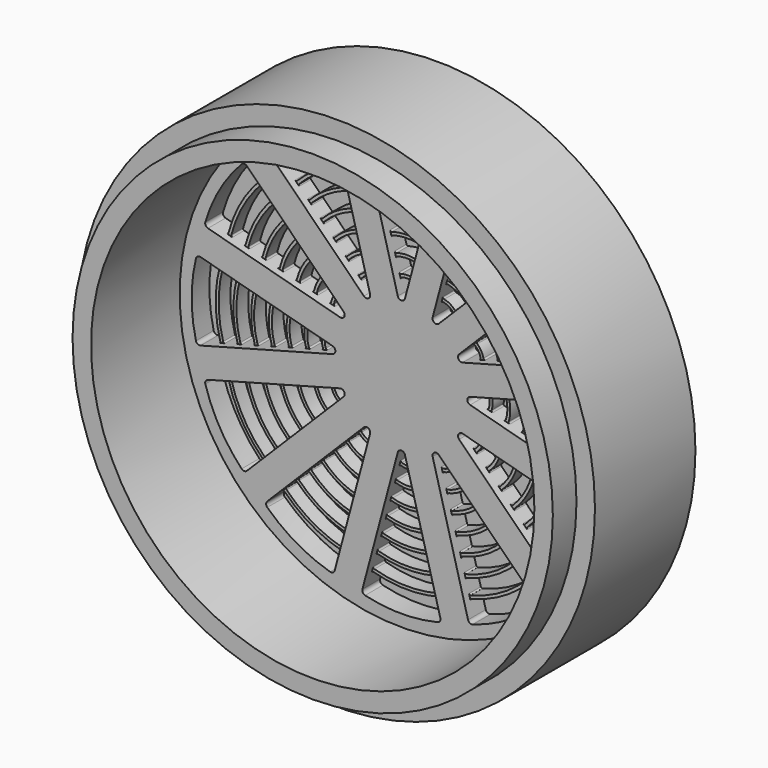
from build123d import *

# Parameters (mm, degrees)
F0_R     = 35
F1_DEPTH = 21
F2_R     = 30
F3_DEPTH = 15
F4_R     = 35
F4_R_2   = 32.5
F5_DEPTH = 4
F7_DEPTH = 3
F9_DEPTH = 2


with BuildPart() as f1:
    # F0 (on Front) → F1 (new body)
    with BuildSketch(Plane.XZ):
        Circle(F0_R)
    extrude(amount=F1_DEPTH)

    # F2 (on face) → F3 (cut)
    with BuildSketch(Plane.XZ.offset(21)):
        Circle(F2_R)
    extrude(amount=-F3_DEPTH, mode=Mode.SUBTRACT)

    # F4 (on face) → F5 (cut)
    with BuildSketch(Plane.XZ.offset(21)):
        Circle(F4_R)
        Circle(F4_R_2, mode=Mode.SUBTRACT)
    extrude(amount=-F5_DEPTH, mode=Mode.SUBTRACT)

    # F6 (on face) → F7 (cut)
    with BuildSketch(Plane.XZ.offset(6)):
        with BuildLine():
            Line((-18.1588429973, 20.9040335257), (-5.0694792169, 7.8146697453))
            ThreePointArc((-5.0694792169, 7.8146697453), (-4.4659258263, 7.735210434), (-4.2329629131, 8.2976326584))
            Line((-4.2329629131, 8.2976326584), (-9.0240025762, 26.1780361019))
            ThreePointArc((-9.0240025762, 26.1780361019), (-9.262295568, 26.4846731704), (-9.6481830883, 26.5282697693))
            ThreePointArc((-9.6481830883, 26.5282697693), (-14.1916572872, 24.5806714651), (-18.1500639945, 21.6197065395))
            ThreePointArc((-18.1500639945, 21.6197065395), (-18.3052519925, 21.2637198445), (-18.1588429973, 20.9040335257))
        make_face()
        with BuildLine():
            Line((-5.2740025762, 27.1828455735), (-0.4829629131, 9.30244213))
            ThreePointArc((-0.4829629131, 9.30244213), (0, 8.9318516526), (0.4829629131, 9.30244213))
            Line((0.4829629131, 9.30244213), (5.2740025762, 27.1828455735))
            ThreePointArc((5.2740025762, 27.1828455735), (5.2209533259, 27.5675475605), (4.9085632298, 27.7982470828))
            ThreePointArc((4.9085632298, 27.7982470828), (0, 28.3833145745), (-4.9085632298, 27.7982470828))
            ThreePointArc((-4.9085632298, 27.7982470828), (-5.2209533259, 27.5675475605), (-5.2740025762, 27.1828455735))
        make_face()
        with BuildLine():
            Line((9.0240025762, 26.1780361019), (4.2329629131, 8.2976326584))
            ThreePointArc((4.2329629131, 8.2976326584), (4.4659258263, 7.735210434), (5.0694792169, 7.8146697453))
            Line((5.0694792169, 7.8146697453), (18.1588429973, 20.9040335257))
            ThreePointArc((18.1588429973, 20.9040335257), (18.3052519925, 21.2637198445), (18.1500639945, 21.6197065395))
            ThreePointArc((18.1500639945, 21.6197065395), (14.1916572872, 24.5806714651), (9.6481830883, 26.5282697693))
            ThreePointArc((9.6481830883, 26.5282697693), (9.262295568, 26.4846731704), (9.0240025762, 26.1780361019))
        make_face()
        with BuildLine():
            Line((20.9040335257, 18.1588429973), (7.8146697453, 5.0694792169))
            ThreePointArc((7.8146697453, 5.0694792169), (7.735210434, 4.4659258263), (8.2976326584, 4.2329629131))
            Line((8.2976326584, 4.2329629131), (26.1780361019, 9.0240025762))
            ThreePointArc((26.1780361019, 9.0240025762), (26.4846731704, 9.262295568), (26.5282697693, 9.6481830883))
            ThreePointArc((26.5282697693, 9.6481830883), (24.5806714651, 14.1916572872), (21.6197065395, 18.1500639945))
            ThreePointArc((21.6197065395, 18.1500639945), (21.2637198445, 18.3052519925), (20.9040335257, 18.1588429973))
        make_face()
        with BuildLine():
            Line((27.1828455735, 5.2740025762), (9.30244213, 0.4829629131))
            ThreePointArc((9.30244213, 0.4829629131), (8.9318516526, 0), (9.30244213, -0.4829629131))
            Line((9.30244213, -0.4829629131), (27.1828455735, -5.2740025762))
            ThreePointArc((27.1828455735, -5.2740025762), (27.5675475605, -5.2209533259), (27.7982470828, -4.9085632298))
            ThreePointArc((27.7982470828, -4.9085632298), (28.3833145745, 0), (27.7982470828, 4.9085632298))
            ThreePointArc((27.7982470828, 4.9085632298), (27.5675475605, 5.2209533259), (27.1828455735, 5.2740025762))
        make_face()
        with BuildLine():
            Line((26.1780361019, -9.0240025762), (8.2976326584, -4.2329629131))
            ThreePointArc((8.2976326584, -4.2329629131), (7.735210434, -4.4659258263), (7.8146697453, -5.0694792169))
            Line((7.8146697453, -5.0694792169), (20.9040335257, -18.1588429973))
            ThreePointArc((20.9040335257, -18.1588429973), (21.2637198445, -18.3052519925), (21.6197065395, -18.1500639945))
            ThreePointArc((21.6197065395, -18.1500639945), (24.5806714651, -14.1916572872), (26.5282697693, -9.6481830883))
            ThreePointArc((26.5282697693, -9.6481830883), (26.4846731704, -9.262295568), (26.1780361019, -9.0240025762))
        make_face()
        with BuildLine():
            Line((18.1588429973, -20.9040335257), (5.0694792169, -7.8146697453))
            ThreePointArc((5.0694792169, -7.8146697453), (4.4659258263, -7.735210434), (4.2329629131, -8.2976326584))
            Line((4.2329629131, -8.2976326584), (9.0240025762, -26.1780361019))
            ThreePointArc((9.0240025762, -26.1780361019), (9.262295568, -26.4846731704), (9.6481830883, -26.5282697693))
            ThreePointArc((9.6481830883, -26.5282697693), (14.1916572872, -24.5806714651), (18.1500639945, -21.6197065395))
            ThreePointArc((18.1500639945, -21.6197065395), (18.3052519925, -21.2637198445), (18.1588429973, -20.9040335257))
        make_face()
        with BuildLine():
            Line((5.2740025762, -27.1828455735), (0.4829629131, -9.30244213))
            ThreePointArc((0.4829629131, -9.30244213), (0, -8.9318516526), (-0.4829629131, -9.30244213))
            Line((-0.4829629131, -9.30244213), (-5.2740025762, -27.1828455735))
            ThreePointArc((-5.2740025762, -27.1828455735), (-5.2209533259, -27.5675475605), (-4.9085632298, -27.7982470828))
            ThreePointArc((-4.9085632298, -27.7982470828), (0, -28.3833145745), (4.9085632298, -27.7982470828))
            ThreePointArc((4.9085632298, -27.7982470828), (5.2209533259, -27.5675475605), (5.2740025762, -27.1828455735))
        make_face()
        with BuildLine():
            Line((-9.0240025762, -26.1780361019), (-4.2329629131, -8.2976326584))
            ThreePointArc((-4.2329629131, -8.2976326584), (-4.4659258263, -7.735210434), (-5.0694792169, -7.8146697453))
            Line((-5.0694792169, -7.8146697453), (-18.1588429973, -20.9040335257))
            ThreePointArc((-18.1588429973, -20.9040335257), (-18.3052519925, -21.2637198445), (-18.1500639945, -21.6197065395))
            ThreePointArc((-18.1500639945, -21.6197065395), (-14.1916572872, -24.5806714651), (-9.6481830883, -26.5282697693))
            ThreePointArc((-9.6481830883, -26.5282697693), (-9.262295568, -26.4846731704), (-9.0240025762, -26.1780361019))
        make_face()
        with BuildLine():
            Line((-20.9040335257, -18.1588429973), (-7.8146697453, -5.0694792169))
            ThreePointArc((-7.8146697453, -5.0694792169), (-7.735210434, -4.4659258263), (-8.2976326584, -4.2329629131))
            Line((-8.2976326584, -4.2329629131), (-26.1780361019, -9.0240025762))
            ThreePointArc((-26.1780361019, -9.0240025762), (-26.4846731704, -9.262295568), (-26.5282697693, -9.6481830883))
            ThreePointArc((-26.5282697693, -9.6481830883), (-24.5806714651, -14.1916572872), (-21.6197065395, -18.1500639945))
            ThreePointArc((-21.6197065395, -18.1500639945), (-21.2637198445, -18.3052519925), (-20.9040335257, -18.1588429973))
        make_face()
        with BuildLine():
            Line((-27.1828455735, -5.2740025762), (-9.30244213, -0.4829629131))
            ThreePointArc((-9.30244213, -0.4829629131), (-8.9318516526, 0), (-9.30244213, 0.4829629131))
            Line((-9.30244213, 0.4829629131), (-27.1828455735, 5.2740025762))
            ThreePointArc((-27.1828455735, 5.2740025762), (-27.5675475605, 5.2209533259), (-27.7982470828, 4.9085632298))
            ThreePointArc((-27.7982470828, 4.9085632298), (-28.3833145745, 0), (-27.7982470828, -4.9085632298))
            ThreePointArc((-27.7982470828, -4.9085632298), (-27.5675475605, -5.2209533259), (-27.1828455735, -5.2740025762))
        make_face()
        with BuildLine():
            Line((-26.1780361019, 9.0240025762), (-8.2976326584, 4.2329629131))
            ThreePointArc((-8.2976326584, 4.2329629131), (-7.735210434, 4.4659258263), (-7.8146697453, 5.0694792169))
            Line((-7.8146697453, 5.0694792169), (-20.9040335257, 18.1588429973))
            ThreePointArc((-20.9040335257, 18.1588429973), (-21.2637198445, 18.3052519925), (-21.6197065395, 18.1500639945))
            ThreePointArc((-21.6197065395, 18.1500639945), (-24.5806714651, 14.1916572872), (-26.5282697693, 9.6481830883))
            ThreePointArc((-26.5282697693, 9.6481830883), (-26.4846731704, 9.262295568), (-26.1780361019, 9.0240025762))
        make_face()
    extrude(amount=-F7_DEPTH, mode=Mode.SUBTRACT)

    # F8 (on face) → F9 (join)
    with BuildSketch(Plane.XZ.offset(3)):
        with BuildLine():
            ThreePointArc((-4.5620923554, 25.3063660221), (-4.7149095825, 25.3253293202), (-4.8089550086, 25.4472644234))
            Line((-4.8089550086, 25.4472644234), (-4.6019142903, 24.6745779436))
            ThreePointArc((-4.6019142903, 24.6745779436), (-4.5824520179, 24.8254394644), (-4.4624998314, 24.9189779671))
            ThreePointArc((-4.4624998314, 24.9189779671), (0, 25.5301079628), (4.4624998314, 24.9189779671))
            ThreePointArc((4.4624998314, 24.9189779671), (4.5824520179, 24.8254394644), (4.6019142903, 24.6745779436))
            Line((4.6019142903, 24.6745779436), (4.8089550086, 25.4472644234))
            ThreePointArc((4.8089550086, 25.4472644234), (4.7149095825, 25.3253293202), (4.5620923554, 25.3063660221))
            ThreePointArc((4.5620923554, 25.3063660221), (0, 25.9300105969), (-4.5620923554, 25.3063660221))
        make_face()
        with BuildLine():
            ThreePointArc((-3.9407532691, 22.988739695), (-4.0937405711, 23.0075367494), (-4.1879257075, 23.1295515187))
            Line((-4.1879257075, 23.1295515187), (-4.1351987777, 22.9327719378))
            Line((-4.1351987777, 22.9327719378), (-4.0316711597, 22.5464016073))
            Line((-4.0316711597, 22.5464016073), (-3.9808902311, 22.3568846019))
            ThreePointArc((-3.9808902311, 22.3568846019), (-3.9615162399, 22.5075912014), (-3.8418191748, 22.6011884411))
            ThreePointArc((-3.8418191748, 22.6011884411), (0, 23.1308073469), (3.8418191748, 22.6011884411))
            ThreePointArc((3.8418191748, 22.6011884411), (3.9615162399, 22.5075912014), (3.9808902311, 22.3568846019))
            Line((3.9808902311, 22.3568846019), (4.0316711597, 22.5464016073))
            Line((4.0316711597, 22.5464016073), (4.1351987777, 22.9327719378))
            Line((4.1351987777, 22.9327719378), (4.1879257075, 23.1295515187))
            ThreePointArc((4.1879257075, 23.1295515187), (4.0937405711, 23.0075367494), (3.9407532691, 22.988739695))
            ThreePointArc((3.9407532691, 22.988739695), (0, 23.5306748163), (-3.9407532691, 22.988739695))
        make_face()
        with BuildLine():
            ThreePointArc((-3.319348466, 20.6713488221), (-3.4725713004, 20.6899146821), (-3.5669503008, 20.8120397508))
            Line((-3.5669503008, 20.8120397508), (-3.5140330695, 20.6145499547))
            Line((-3.5140330695, 20.6145499547), (-3.4105054514, 20.2281796242))
            Line((-3.4105054514, 20.2281796242), (-3.3599235163, 20.0394052724))
            ThreePointArc((-3.3599235163, 20.0394052724), (-3.3406740766, 20.1898927533), (-3.2213375727, 20.2835721089))
            ThreePointArc((-3.2213375727, 20.2835721089), (0, 20.7317911896), (3.2213375727, 20.2835721089))
            ThreePointArc((3.2213375727, 20.2835721089), (3.3406740766, 20.1898927533), (3.3599235163, 20.0394052724))
            Line((3.3599235163, 20.0394052724), (3.4105054514, 20.2281796242))
            Line((3.4105054514, 20.2281796242), (3.5140330695, 20.6145499547))
            Line((3.5140330695, 20.6145499547), (3.5669503008, 20.8120397508))
            ThreePointArc((3.5669503008, 20.8120397508), (3.4725713004, 20.6899146821), (3.319348466, 20.6713488221))
            ThreePointArc((3.319348466, 20.6713488221), (0, 21.1316003398), (-3.319348466, 20.6713488221))
        make_face()
        with BuildLine():
            ThreePointArc((-2.6978319486, 18.3543672974), (-2.8514025291, 18.3725897474), (-2.9460685756, 18.4948776066))
            Line((-2.9460685756, 18.4948776066), (-2.8928673612, 18.2963279716))
            Line((-2.8928673612, 18.2963279716), (-2.7893397432, 17.9099576411))
            Line((-2.7893397432, 17.9099576411), (-2.7390577856, 17.7223028208))
            ThreePointArc((-2.7390577856, 17.7223028208), (-2.719997277, 17.87245669), (-2.6012091026, 17.9662589131))
            ThreePointArc((-2.6012091026, 17.9662589131), (0, 18.3332772543), (2.6012091026, 17.9662589131))
            ThreePointArc((2.6012091026, 17.9662589131), (2.719997277, 17.87245669), (2.7390577856, 17.7223028208))
            Line((2.7390577856, 17.7223028208), (2.7893397432, 17.9099576411))
            Line((2.7893397432, 17.9099576411), (2.8928673612, 18.2963279716))
            Line((2.8928673612, 18.2963279716), (2.9460685756, 18.4948776066))
            ThreePointArc((2.9460685756, 18.4948776066), (2.8514025291, 18.3725897474), (2.6978319486, 18.3543672974))
            ThreePointArc((2.6978319486, 18.3543672974), (0, 18.732979052), (-2.6978319486, 18.3543672974))
        make_face()
        with BuildLine():
            ThreePointArc((-2.0761019645, 16.0381959448), (-2.2302376242, 16.0558550494), (-2.3253722264, 16.1784072955))
            Line((-2.3253722264, 16.1784072955), (-2.271701653, 15.9781059885))
            Line((-2.271701653, 15.9781059885), (-2.1681740349, 15.591735658))
            Line((-2.1681740349, 15.591735658), (-2.1183959599, 15.4059613529))
            ThreePointArc((-2.1183959599, 15.4059613529), (-2.0996559784, 15.5555458032), (-1.9818019363, 15.6495517573))
            ThreePointArc((-1.9818019363, 15.6495517573), (0, 15.9357815217), (1.9818019363, 15.6495517573))
            ThreePointArc((1.9818019363, 15.6495517573), (2.0996559784, 15.5555458032), (2.1183959599, 15.4059613529))
            Line((2.1183959599, 15.4059613529), (2.1681740349, 15.591735658))
            Line((2.1681740349, 15.591735658), (2.271701653, 15.9781059885))
            Line((2.271701653, 15.9781059885), (2.3253722264, 16.1784072955))
            ThreePointArc((2.3253722264, 16.1784072955), (2.2302376242, 16.0558550494), (2.0761019645, 16.0381959448))
            ThreePointArc((2.0761019645, 16.0381959448), (0, 16.3352514504), (-2.0761019645, 16.0381959448))
        make_face()
        with BuildLine():
            ThreePointArc((-1.4538810303, 13.7240107468), (-1.6090945281, 13.7405767627), (-1.7051302794, 13.8636328363))
            Line((-1.7051302794, 13.8636328363), (-1.6505359447, 13.6598840054))
            Line((-1.6505359447, 13.6598840054), (-1.5470083267, 13.2735136749))
            Line((-1.5470083267, 13.2735136749), (-1.4982523683, 13.0915539612))
            ThreePointArc((-1.4982523683, 13.0915539612), (-1.4801747728, 13.2399476777), (-1.3642667907, 13.3343554859))
            ThreePointArc((-1.3642667907, 13.3343554859), (0, 13.5408931884), (1.3642667907, 13.3343554859))
            ThreePointArc((1.3642667907, 13.3343554859), (1.4801747728, 13.2399476777), (1.4982523683, 13.0915539612))
            Line((1.4982523683, 13.0915539612), (1.5470083267, 13.2735136749))
            Line((1.5470083267, 13.2735136749), (1.6505359447, 13.6598840054))
            Line((1.6505359447, 13.6598840054), (1.7051302794, 13.8636328363))
            ThreePointArc((1.7051302794, 13.8636328363), (1.6090945281, 13.7405767627), (1.4538810303, 13.7240107468))
            ThreePointArc((1.4538810303, 13.7240107468), (0, 13.9397013742), (-1.4538810303, 13.7240107468))
        make_face()
        with BuildLine():
            ThreePointArc((-0.8300754785, 11.4173624254), (-0.9881428083, 11.430911726), (-1.0866141602, 11.5552992541))
            Line((-1.0866141602, 11.5552992541), (-1.0293702365, 11.3416620223))
            Line((-1.0293702365, 11.3416620223), (-0.9258426184, 10.9552916918))
            Line((-0.9258426184, 10.9552916918), (-0.8802591635, 10.7851719219))
            ThreePointArc((-0.8802591635, 10.7851719219), (-0.864340569, 10.9295454651), (-0.7549266143, 11.0250740377))
            ThreePointArc((-0.7549266143, 11.0250740377), (0, 11.1570469578), (0.7549266143, 11.0250740377))
            ThreePointArc((0.7549266143, 11.0250740377), (0.864340569, 10.9295454651), (0.8802591635, 10.7851719219))
            Line((0.8802591635, 10.7851719219), (0.9258426184, 10.9552916918))
            Line((0.9258426184, 10.9552916918), (1.0293702365, 11.3416620223))
            Line((1.0293702365, 11.3416620223), (1.0866141602, 11.5552992541))
            ThreePointArc((1.0866141602, 11.5552992541), (0.9881428083, 11.430911726), (0.8300754785, 11.4173624254))
            ThreePointArc((0.8300754785, 11.4173624254), (0, 11.5523075484), (-0.8300754785, 11.4173624254))
        make_face()
        with BuildLine():
            Line((8.5589550086, 24.4424549518), (8.3519142903, 23.6697684719))
            ThreePointArc((8.3519142903, 23.6697684719), (8.4441998731, 23.7906872453), (8.5948507651, 23.8117178716))
            ThreePointArc((8.5948507651, 23.8117178716), (12.7650539814, 22.1097220572), (16.3241272019, 19.3492180401))
            ThreePointArc((16.3241272019, 19.3492180401), (16.3812395914, 19.2082352273), (16.3226636532, 19.0678541816))
            Line((16.3226636532, 19.0678541816), (16.8883094148, 19.6334999432))
            ThreePointArc((16.8883094148, 19.6334999432), (16.7458961351, 19.5749237592), (16.6040708853, 19.6349096749))
            ThreePointArc((16.6040708853, 19.6349096749), (12.9650052985, 22.4560478973), (8.7022951368, 24.1970020303))
            ThreePointArc((8.7022951368, 24.1970020303), (8.5794331851, 24.2898333417), (8.5589550086, 24.4424549518))
        make_face()
        with BuildLine():
            Line((7.7816711597, 21.5415921357), (7.7308902311, 21.3520751303))
            ThreePointArc((7.7308902311, 21.3520751303), (7.8230218995, 21.4729038783), (7.9734812184, 21.4941129331))
            ThreePointArc((7.9734812184, 21.4941129331), (11.5654036734, 20.0318667724), (14.6277072226, 17.6522937583))
            ThreePointArc((14.6277072226, 17.6522937583), (14.6845693019, 17.5113876385), (14.6259943708, 17.3711848991))
            Line((14.6259943708, 17.3711848991), (14.7647304476, 17.509920976))
            Line((14.7647304476, 17.509920976), (15.0475731601, 17.7927636885))
            Line((15.0475731601, 17.7927636885), (15.1916258112, 17.9368163396))
            ThreePointArc((15.1916258112, 17.9368163396), (15.0490517058, 17.8782410179), (14.9071622886, 17.9384559423))
            ThreePointArc((14.9071622886, 17.9384559423), (11.7653374081, 20.3781621591), (8.0815774064, 21.8792092114))
            ThreePointArc((8.0815774064, 21.8792092114), (7.9584850436, 21.9719815891), (7.9379257075, 22.1247420471))
            Line((7.9379257075, 22.1247420471), (7.8851987777, 21.9279624662))
            Line((7.8851987777, 21.9279624662), (7.7816711597, 21.5415921357))
        make_face()
        with BuildLine():
            Line((7.1605054514, 19.2233701526), (7.1099235163, 19.0345958008))
            ThreePointArc((7.1099235163, 19.0345958008), (7.2018377606, 19.1552970623), (7.3520258823, 19.1767575122))
            ThreePointArc((7.3520258823, 19.1767575122), (10.3658955948, 17.9542578361), (12.9315462266, 15.9554199395))
            ThreePointArc((12.9315462266, 15.9554199395), (12.9880549927, 15.8146229857), (12.9294817561, 15.6746722845))
            Line((12.9294817561, 15.6746722845), (13.0676741728, 15.8128647012))
            Line((13.0676741728, 15.8128647012), (13.3505168852, 16.0957074136))
            Line((13.3505168852, 16.0957074136), (13.49508945, 16.2402799783))
            ThreePointArc((13.49508945, 16.2402799783), (13.3522923036, 16.1817060666), (13.2103145066, 16.2422389774))
            ThreePointArc((13.2103145066, 16.2422389774), (10.5658001699, 18.3005027169), (7.4610343155, 19.5615874434))
            ThreePointArc((7.4610343155, 19.5615874434), (7.3376223785, 19.654277367), (7.3169503008, 19.8072302792))
            Line((7.3169503008, 19.8072302792), (7.2640330695, 19.6097404831))
            Line((7.2640330695, 19.6097404831), (7.1605054514, 19.2233701526))
        make_face()
        with BuildLine():
            Line((6.5393397432, 16.9051481695), (6.4890577856, 16.7174933492))
            ThreePointArc((6.4890577856, 16.7174933492), (6.5806416049, 16.8380001601), (6.7304162932, 16.859841181))
            ThreePointArc((6.7304162932, 16.859841181), (9.1666386271, 15.8770838368), (11.2358426199, 14.2586320784))
            ThreePointArc((11.2358426199, 14.2586320784), (11.2918150851, 14.1180028831), (11.2332450352, 13.9784355636))
            Line((11.2332450352, 13.9784355636), (11.3706178979, 14.1158084263))
            Line((11.3706178979, 14.1158084263), (11.6534606104, 14.3986511388))
            Line((11.6534606104, 14.3986511388), (11.7988090311, 14.5439995594))
            ThreePointArc((11.7988090311, 14.5439995594), (11.6556819003, 14.48542819), (11.5135746513, 14.5464323756))
            ThreePointArc((11.5135746513, 14.5464323756), (9.366489526, 16.2232357476), (6.840792646, 17.2442643242))
            ThreePointArc((6.840792646, 17.2442643242), (6.7169078471, 17.3368307191), (6.6960685756, 17.490068135))
            Line((6.6960685756, 17.490068135), (6.6428673612, 17.2915185))
            Line((6.6428673612, 17.2915185), (6.5393397432, 16.9051481695))
        make_face()
        with BuildLine():
            Line((5.9181740349, 14.5869261864), (5.8683959599, 14.4011518813))
            ThreePointArc((5.8683959599, 14.4011518813), (5.959417485, 14.5213258245), (6.1084850566, 14.5438103478))
            ThreePointArc((6.1084850566, 14.5438103478), (7.9678907608, 13.8007916269), (9.5410667007, 12.5620084115))
            ThreePointArc((9.5410667007, 12.5620084115), (9.5961283181, 12.421669846), (9.537565393, 12.2827559214))
            Line((9.537565393, 12.2827559214), (9.6735616231, 12.4187521515))
            Line((9.6735616231, 12.4187521515), (9.9564043355, 12.7015948639))
            Line((9.9564043355, 12.7015948639), (10.1030350691, 12.8482255974))
            ThreePointArc((10.1030350691, 12.8482255974), (9.9593699637, 12.7896595401), (9.8170550145, 12.8514341368))
            ThreePointArc((9.8170550145, 12.8514341368), (8.1676257252, 14.1467427333), (6.2211409303, 14.9275361013))
            ThreePointArc((6.2211409303, 14.9275361013), (6.0964850856, 15.0198971643), (6.0753722264, 15.1735978239))
            Line((6.0753722264, 15.1735978239), (6.021701653, 14.9732965169))
            Line((6.021701653, 14.9732965169), (5.9181740349, 14.5869261864))
        make_face()
        with BuildLine():
            ThreePointArc((5.2482523683, 12.0867444896), (5.3381048836, 12.2062184201), (5.4856880447, 12.2300239893))
            ThreePointArc((5.4856880447, 12.2300239893), (6.7704465942, 11.7267574911), (7.8486674412, 10.8657571986))
            ThreePointArc((7.8486674412, 10.8657571986), (7.9018427942, 10.7260436473), (7.8433015929, 10.5884921212))
            Line((7.8433015929, 10.5884921212), (7.9765053482, 10.7216958766))
            Line((7.9765053482, 10.7216958766), (8.2593480607, 11.0045385891))
            Line((8.2593480607, 11.0045385891), (8.4085025569, 11.1536930853))
            ThreePointArc((8.4085025569, 11.1536930853), (8.2638051198, 11.0951412751), (8.1211032797, 11.1584014334))
            ThreePointArc((8.1211032797, 11.1584014334), (6.9698506871, 12.0721355112), (5.602907467, 12.6122824637))
            ThreePointArc((5.602907467, 12.6122824637), (5.4767716429, 12.7042358032), (5.4551302794, 12.8588233647))
            Line((5.4551302794, 12.8588233647), (5.4005359447, 12.6550745338))
            Line((5.4005359447, 12.6550745338), (5.2970083267, 12.2687042033))
            Line((5.2970083267, 12.2687042033), (5.2482523683, 12.0867444896))
        make_face()
        with BuildLine():
            ThreePointArc((4.9898147613, 10.3027636439), (4.8596990885, 10.3935313473), (4.8366141602, 10.5504897825))
            Line((4.8366141602, 10.5504897825), (4.7793702365, 10.3368525507))
            Line((4.7793702365, 10.3368525507), (4.6758426184, 9.9504822202))
            Line((4.6758426184, 9.9504822202), (4.6302591635, 9.7803624502))
            ThreePointArc((4.6302591635, 9.7803624502), (4.7162318423, 9.8974343091), (4.8587513928, 9.9254575024))
            ThreePointArc((4.8587513928, 9.9254575024), (5.5785234789, 9.6622860967), (6.1663226448, 9.1705308881))
            ThreePointArc((6.1663226448, 9.1705308881), (6.2133136228, 9.0330937401), (6.1549127584, 8.9001032868))
            Line((6.1549127584, 8.9001032868), (6.2794490734, 9.0246396018))
            Line((6.2794490734, 9.0246396018), (6.5622917859, 9.3074823142))
            Line((6.5622917859, 9.3074823142), (6.7186850939, 9.4638756223))
            ThreePointArc((6.7186850939, 9.4638756223), (6.5712126376, 9.405388539), (6.4275476642, 9.4726881654))
            ThreePointArc((6.4275476642, 9.4726881654), (5.7761537742, 10.0045918092), (4.9898147613, 10.3027636439))
        make_face()
        with BuildLine():
            ThreePointArc((9.4726881654, 6.4275476642), (9.405388539, 6.5712126376), (9.4638756223, 6.7186850939))
            Line((9.4638756223, 6.7186850939), (9.3074823142, 6.5622917859))
            Line((9.3074823142, 6.5622917859), (9.0246396018, 6.2794490734))
            Line((9.0246396018, 6.2794490734), (8.9001032868, 6.1549127584))
            ThreePointArc((8.9001032868, 6.1549127584), (9.0330937401, 6.2133136228), (9.1705308881, 6.1663226448))
            ThreePointArc((9.1705308881, 6.1663226448), (9.6622860967, 5.5785234789), (9.9254575024, 4.8587513928))
            ThreePointArc((9.9254575024, 4.8587513928), (9.8974343091, 4.7162318423), (9.7803624502, 4.6302591635))
            Line((9.7803624502, 4.6302591635), (9.9504822202, 4.6758426184))
            Line((9.9504822202, 4.6758426184), (10.3368525507, 4.7793702365))
            Line((10.3368525507, 4.7793702365), (10.5504897825, 4.8366141602))
            ThreePointArc((10.5504897825, 4.8366141602), (10.3935313473, 4.8596990885), (10.3027636439, 4.9898147613))
            ThreePointArc((10.3027636439, 4.9898147613), (10.0045918092, 5.7761537742), (9.4726881654, 6.4275476642))
        make_face()
        with BuildLine():
            ThreePointArc((10.5884921212, 7.8433015929), (10.7260436473, 7.9018427942), (10.8657571986, 7.8486674412))
            ThreePointArc((10.8657571986, 7.8486674412), (11.7267574911, 6.7704465942), (12.2300239893, 5.4856880447))
            ThreePointArc((12.2300239893, 5.4856880447), (12.2062184201, 5.3381048836), (12.0867444896, 5.2482523683))
            Line((12.0867444896, 5.2482523683), (12.2687042033, 5.2970083267))
            Line((12.2687042033, 5.2970083267), (12.6550745338, 5.4005359447))
            Line((12.6550745338, 5.4005359447), (12.8588233647, 5.4551302794))
            ThreePointArc((12.8588233647, 5.4551302794), (12.7042358032, 5.4767716429), (12.6122824637, 5.602907467))
            ThreePointArc((12.6122824637, 5.602907467), (12.0721355112, 6.9698506871), (11.1584014334, 8.1211032797))
            ThreePointArc((11.1584014334, 8.1211032797), (11.0951412751, 8.2638051198), (11.1536930853, 8.4085025569))
            Line((11.1536930853, 8.4085025569), (11.0045385891, 8.2593480607))
            Line((11.0045385891, 8.2593480607), (10.7216958766, 7.9765053482))
            Line((10.7216958766, 7.9765053482), (10.5884921212, 7.8433015929))
        make_face()
        with BuildLine():
            Line((12.4187521515, 9.6735616231), (12.2827559214, 9.537565393))
            ThreePointArc((12.2827559214, 9.537565393), (12.421669846, 9.5961283181), (12.5620084115, 9.5410667007))
            ThreePointArc((12.5620084115, 9.5410667007), (13.8007916269, 7.9678907608), (14.5438103478, 6.1084850566))
            ThreePointArc((14.5438103478, 6.1084850566), (14.5213258245, 5.959417485), (14.4011518813, 5.8683959599))
            Line((14.4011518813, 5.8683959599), (14.5869261864, 5.9181740349))
            Line((14.5869261864, 5.9181740349), (14.9732965169, 6.021701653))
            Line((14.9732965169, 6.021701653), (15.1735978239, 6.0753722264))
            ThreePointArc((15.1735978239, 6.0753722264), (15.0198971643, 6.0964850856), (14.9275361013, 6.2211409303))
            ThreePointArc((14.9275361013, 6.2211409303), (14.1467427333, 8.1676257252), (12.8514341368, 9.8170550145))
            ThreePointArc((12.8514341368, 9.8170550145), (12.7896595401, 9.9593699637), (12.8482255974, 10.1030350691))
            Line((12.8482255974, 10.1030350691), (12.7015948639, 9.9564043355))
            Line((12.7015948639, 9.9564043355), (12.4187521515, 9.6735616231))
        make_face()
        with BuildLine():
            Line((14.1158084263, 11.3706178979), (13.9784355636, 11.2332450352))
            ThreePointArc((13.9784355636, 11.2332450352), (14.1180028831, 11.2918150851), (14.2586320784, 11.2358426199))
            ThreePointArc((14.2586320784, 11.2358426199), (15.8770838368, 9.1666386271), (16.859841181, 6.7304162932))
            ThreePointArc((16.859841181, 6.7304162932), (16.8380001601, 6.5806416049), (16.7174933492, 6.4890577856))
            Line((16.7174933492, 6.4890577856), (16.9051481695, 6.5393397432))
            Line((16.9051481695, 6.5393397432), (17.2915185, 6.6428673612))
            Line((17.2915185, 6.6428673612), (17.490068135, 6.6960685756))
            ThreePointArc((17.490068135, 6.6960685756), (17.3368307191, 6.7169078471), (17.2442643242, 6.840792646))
            ThreePointArc((17.2442643242, 6.840792646), (16.2232357476, 9.366489526), (14.5464323756, 11.5135746513))
            ThreePointArc((14.5464323756, 11.5135746513), (14.48542819, 11.6556819003), (14.5439995594, 11.7988090311))
            Line((14.5439995594, 11.7988090311), (14.3986511388, 11.6534606104))
            Line((14.3986511388, 11.6534606104), (14.1158084263, 11.3706178979))
        make_face()
        with BuildLine():
            Line((15.8128647012, 13.0676741728), (15.6746722845, 12.9294817561))
            ThreePointArc((15.6746722845, 12.9294817561), (15.8146229857, 12.9880549927), (15.9554199395, 12.9315462266))
            ThreePointArc((15.9554199395, 12.9315462266), (17.9542578361, 10.3658955948), (19.1767575122, 7.3520258823))
            ThreePointArc((19.1767575122, 7.3520258823), (19.1552970623, 7.2018377606), (19.0345958008, 7.1099235163))
            Line((19.0345958008, 7.1099235163), (19.2233701526, 7.1605054514))
            Line((19.2233701526, 7.1605054514), (19.6097404831, 7.2640330695))
            Line((19.6097404831, 7.2640330695), (19.8072302792, 7.3169503008))
            ThreePointArc((19.8072302792, 7.3169503008), (19.654277367, 7.3376223785), (19.5615874434, 7.4610343155))
            ThreePointArc((19.5615874434, 7.4610343155), (18.3005027169, 10.5658001699), (16.2422389774, 13.2103145066))
            ThreePointArc((16.2422389774, 13.2103145066), (16.1817060666, 13.3522923036), (16.2402799783, 13.49508945))
            Line((16.2402799783, 13.49508945), (16.0957074136, 13.3505168852))
            Line((16.0957074136, 13.3505168852), (15.8128647012, 13.0676741728))
        make_face()
        with BuildLine():
            Line((17.509920976, 14.7647304476), (17.3711848991, 14.6259943708))
            ThreePointArc((17.3711848991, 14.6259943708), (17.5113876385, 14.6845693019), (17.6522937583, 14.6277072226))
            ThreePointArc((17.6522937583, 14.6277072226), (20.0318667724, 11.5654036734), (21.4941129331, 7.9734812184))
            ThreePointArc((21.4941129331, 7.9734812184), (21.4729038783, 7.8230218995), (21.3520751303, 7.7308902311))
            Line((21.3520751303, 7.7308902311), (21.5415921357, 7.7816711597))
            Line((21.5415921357, 7.7816711597), (21.9279624662, 7.8851987777))
            Line((21.9279624662, 7.8851987777), (22.1247420471, 7.9379257075))
            ThreePointArc((22.1247420471, 7.9379257075), (21.9719815891, 7.9584850436), (21.8792092114, 8.0815774064))
            ThreePointArc((21.8792092114, 8.0815774064), (20.3781621591, 11.7653374081), (17.9384559423, 14.9071622886))
            ThreePointArc((17.9384559423, 14.9071622886), (17.8782410179, 15.0490517058), (17.9368163396, 15.1916258112))
            Line((17.9368163396, 15.1916258112), (17.7927636885, 15.0475731601))
            Line((17.7927636885, 15.0475731601), (17.509920976, 14.7647304476))
        make_face()
        with BuildLine():
            Line((19.6334999432, 16.8883094148), (19.0678541816, 16.3226636532))
            ThreePointArc((19.0678541816, 16.3226636532), (19.2082352273, 16.3812395914), (19.3492180401, 16.3241272019))
            ThreePointArc((19.3492180401, 16.3241272019), (22.1097220572, 12.7650539814), (23.8117178716, 8.5948507651))
            ThreePointArc((23.8117178716, 8.5948507651), (23.7906872453, 8.4441998731), (23.6697684719, 8.3519142903))
            Line((23.6697684719, 8.3519142903), (24.4424549518, 8.5589550086))
            ThreePointArc((24.4424549518, 8.5589550086), (24.2898333417, 8.5794331851), (24.1970020303, 8.7022951368))
            ThreePointArc((24.1970020303, 8.7022951368), (22.4560478973, 12.9650052985), (19.6349096749, 16.6040708853))
            ThreePointArc((19.6349096749, 16.6040708853), (19.5749237592, 16.7458961351), (19.6334999432, 16.8883094148))
        make_face()
        with BuildLine():
            ThreePointArc((11.4173624254, 0.8300754785), (11.430911726, 0.9881428083), (11.5552992541, 1.0866141602))
            Line((11.5552992541, 1.0866141602), (11.3416620223, 1.0293702365))
            Line((11.3416620223, 1.0293702365), (10.9552916918, 0.9258426184))
            Line((10.9552916918, 0.9258426184), (10.7851719219, 0.8802591635))
            ThreePointArc((10.7851719219, 0.8802591635), (10.9295454651, 0.864340569), (11.0250740377, 0.7549266143))
            ThreePointArc((11.0250740377, 0.7549266143), (11.1570469578, 0), (11.0250740377, -0.7549266143))
            ThreePointArc((11.0250740377, -0.7549266143), (10.9295454651, -0.864340569), (10.7851719219, -0.8802591635))
            Line((10.7851719219, -0.8802591635), (10.9552916918, -0.9258426184))
            Line((10.9552916918, -0.9258426184), (11.3416620223, -1.0293702365))
            Line((11.3416620223, -1.0293702365), (11.5552992541, -1.0866141602))
            ThreePointArc((11.5552992541, -1.0866141602), (11.430911726, -0.9881428083), (11.4173624254, -0.8300754785))
            ThreePointArc((11.4173624254, -0.8300754785), (11.5523075484, 0), (11.4173624254, 0.8300754785))
        make_face()
        with BuildLine():
            ThreePointArc((13.0915539612, 1.4982523683), (13.2399476777, 1.4801747728), (13.3343554859, 1.3642667907))
            ThreePointArc((13.3343554859, 1.3642667907), (13.5408931884, 0), (13.3343554859, -1.3642667907))
            ThreePointArc((13.3343554859, -1.3642667907), (13.2399476777, -1.4801747728), (13.0915539612, -1.4982523683))
            Line((13.0915539612, -1.4982523683), (13.2735136749, -1.5470083267))
            Line((13.2735136749, -1.5470083267), (13.6598840054, -1.6505359447))
            Line((13.6598840054, -1.6505359447), (13.8636328363, -1.7051302794))
            ThreePointArc((13.8636328363, -1.7051302794), (13.7405767627, -1.6090945281), (13.7240107468, -1.4538810303))
            ThreePointArc((13.7240107468, -1.4538810303), (13.9397013742, 0), (13.7240107468, 1.4538810303))
            ThreePointArc((13.7240107468, 1.4538810303), (13.7405767627, 1.6090945281), (13.8636328363, 1.7051302794))
            Line((13.8636328363, 1.7051302794), (13.6598840054, 1.6505359447))
            Line((13.6598840054, 1.6505359447), (13.2735136749, 1.5470083267))
            Line((13.2735136749, 1.5470083267), (13.0915539612, 1.4982523683))
        make_face()
        with BuildLine():
            Line((15.591735658, 2.1681740349), (15.4059613529, 2.1183959599))
            ThreePointArc((15.4059613529, 2.1183959599), (15.5555458032, 2.0996559784), (15.6495517573, 1.9818019363))
            ThreePointArc((15.6495517573, 1.9818019363), (15.9357815217, 0), (15.6495517573, -1.9818019363))
            ThreePointArc((15.6495517573, -1.9818019363), (15.5555458032, -2.0996559784), (15.4059613529, -2.1183959599))
            Line((15.4059613529, -2.1183959599), (15.591735658, -2.1681740349))
            Line((15.591735658, -2.1681740349), (15.9781059885, -2.271701653))
            Line((15.9781059885, -2.271701653), (16.1784072955, -2.3253722264))
            ThreePointArc((16.1784072955, -2.3253722264), (16.0558550494, -2.2302376242), (16.0381959448, -2.0761019645))
            ThreePointArc((16.0381959448, -2.0761019645), (16.3352514504, 0), (16.0381959448, 2.0761019645))
            ThreePointArc((16.0381959448, 2.0761019645), (16.0558550494, 2.2302376242), (16.1784072955, 2.3253722264))
            Line((16.1784072955, 2.3253722264), (15.9781059885, 2.271701653))
            Line((15.9781059885, 2.271701653), (15.591735658, 2.1681740349))
        make_face()
        with BuildLine():
            Line((17.9099576411, 2.7893397432), (17.7223028208, 2.7390577856))
            ThreePointArc((17.7223028208, 2.7390577856), (17.87245669, 2.719997277), (17.9662589131, 2.6012091026))
            ThreePointArc((17.9662589131, 2.6012091026), (18.3332772543, 0), (17.9662589131, -2.6012091026))
            ThreePointArc((17.9662589131, -2.6012091026), (17.87245669, -2.719997277), (17.7223028208, -2.7390577856))
            Line((17.7223028208, -2.7390577856), (17.9099576411, -2.7893397432))
            Line((17.9099576411, -2.7893397432), (18.2963279716, -2.8928673612))
            Line((18.2963279716, -2.8928673612), (18.4948776066, -2.9460685756))
            ThreePointArc((18.4948776066, -2.9460685756), (18.3725897474, -2.8514025291), (18.3543672974, -2.6978319486))
            ThreePointArc((18.3543672974, -2.6978319486), (18.732979052, 0), (18.3543672974, 2.6978319486))
            ThreePointArc((18.3543672974, 2.6978319486), (18.3725897474, 2.8514025291), (18.4948776066, 2.9460685756))
            Line((18.4948776066, 2.9460685756), (18.2963279716, 2.8928673612))
            Line((18.2963279716, 2.8928673612), (17.9099576411, 2.7893397432))
        make_face()
        with BuildLine():
            Line((20.2281796242, 3.4105054514), (20.0394052724, 3.3599235163))
            ThreePointArc((20.0394052724, 3.3599235163), (20.1898927533, 3.3406740766), (20.2835721089, 3.2213375727))
            ThreePointArc((20.2835721089, 3.2213375727), (20.7317911896, 0), (20.2835721089, -3.2213375727))
            ThreePointArc((20.2835721089, -3.2213375727), (20.1898927533, -3.3406740766), (20.0394052724, -3.3599235163))
            Line((20.0394052724, -3.3599235163), (20.2281796242, -3.4105054514))
            Line((20.2281796242, -3.4105054514), (20.6145499547, -3.5140330695))
            Line((20.6145499547, -3.5140330695), (20.8120397508, -3.5669503008))
            ThreePointArc((20.8120397508, -3.5669503008), (20.6899146821, -3.4725713004), (20.6713488221, -3.319348466))
            ThreePointArc((20.6713488221, -3.319348466), (21.1316003398, 0), (20.6713488221, 3.319348466))
            ThreePointArc((20.6713488221, 3.319348466), (20.6899146821, 3.4725713004), (20.8120397508, 3.5669503008))
            Line((20.8120397508, 3.5669503008), (20.6145499547, 3.5140330695))
            Line((20.6145499547, 3.5140330695), (20.2281796242, 3.4105054514))
        make_face()
        with BuildLine():
            Line((22.5464016073, 4.0316711597), (22.3568846019, 3.9808902311))
            ThreePointArc((22.3568846019, 3.9808902311), (22.5075912014, 3.9615162399), (22.6011884411, 3.8418191748))
            ThreePointArc((22.6011884411, 3.8418191748), (23.1308073469, 0), (22.6011884411, -3.8418191748))
            ThreePointArc((22.6011884411, -3.8418191748), (22.5075912014, -3.9615162399), (22.3568846019, -3.9808902311))
            Line((22.3568846019, -3.9808902311), (22.5464016073, -4.0316711597))
            Line((22.5464016073, -4.0316711597), (22.9327719378, -4.1351987777))
            Line((22.9327719378, -4.1351987777), (23.1295515187, -4.1879257075))
            ThreePointArc((23.1295515187, -4.1879257075), (23.0075367494, -4.0937405711), (22.988739695, -3.9407532691))
            ThreePointArc((22.988739695, -3.9407532691), (23.5306748163, 0), (22.988739695, 3.9407532691))
            ThreePointArc((22.988739695, 3.9407532691), (23.0075367494, 4.0937405711), (23.1295515187, 4.1879257075))
            Line((23.1295515187, 4.1879257075), (22.9327719378, 4.1351987777))
            Line((22.9327719378, 4.1351987777), (22.5464016073, 4.0316711597))
        make_face()
        with BuildLine():
            Line((25.4472644234, 4.8089550086), (24.6745779436, 4.6019142903))
            ThreePointArc((24.6745779436, 4.6019142903), (24.8254394644, 4.5824520179), (24.9189779671, 4.4624998314))
            ThreePointArc((24.9189779671, 4.4624998314), (25.5301079628, 0), (24.9189779671, -4.4624998314))
            ThreePointArc((24.9189779671, -4.4624998314), (24.8254394644, -4.5824520179), (24.6745779436, -4.6019142903))
            Line((24.6745779436, -4.6019142903), (25.4472644234, -4.8089550086))
            ThreePointArc((25.4472644234, -4.8089550086), (25.3253293202, -4.7149095825), (25.3063660221, -4.5620923554))
            ThreePointArc((25.3063660221, -4.5620923554), (25.9300105969, 0), (25.3063660221, 4.5620923554))
            ThreePointArc((25.3063660221, 4.5620923554), (25.3253293202, 4.7149095825), (25.4472644234, 4.8089550086))
        make_face()
        with BuildLine():
            ThreePointArc((10.3027636439, -4.9898147613), (10.3935313473, -4.8596990885), (10.5504897825, -4.8366141602))
            Line((10.5504897825, -4.8366141602), (10.3368525507, -4.7793702365))
            Line((10.3368525507, -4.7793702365), (9.9504822202, -4.6758426184))
            Line((9.9504822202, -4.6758426184), (9.7803624502, -4.6302591635))
            ThreePointArc((9.7803624502, -4.6302591635), (9.8974343091, -4.7162318423), (9.9254575024, -4.8587513928))
            ThreePointArc((9.9254575024, -4.8587513928), (9.6622860967, -5.5785234789), (9.1705308881, -6.1663226448))
            ThreePointArc((9.1705308881, -6.1663226448), (9.0330937401, -6.2133136228), (8.9001032868, -6.1549127584))
            Line((8.9001032868, -6.1549127584), (9.0246396018, -6.2794490734))
            Line((9.0246396018, -6.2794490734), (9.3074823142, -6.5622917859))
            Line((9.3074823142, -6.5622917859), (9.4638756223, -6.7186850939))
            ThreePointArc((9.4638756223, -6.7186850939), (9.405388539, -6.5712126376), (9.4726881654, -6.4275476642))
            ThreePointArc((9.4726881654, -6.4275476642), (10.0045918092, -5.7761537742), (10.3027636439, -4.9898147613))
        make_face()
        with BuildLine():
            ThreePointArc((12.0867444896, -5.2482523683), (12.2062184201, -5.3381048836), (12.2300239893, -5.4856880447))
            ThreePointArc((12.2300239893, -5.4856880447), (11.7267574911, -6.7704465942), (10.8657571986, -7.8486674412))
            ThreePointArc((10.8657571986, -7.8486674412), (10.7260436473, -7.9018427942), (10.5884921212, -7.8433015929))
            Line((10.5884921212, -7.8433015929), (10.7216958766, -7.9765053482))
            Line((10.7216958766, -7.9765053482), (11.0045385891, -8.2593480607))
            Line((11.0045385891, -8.2593480607), (11.1536930853, -8.4085025569))
            ThreePointArc((11.1536930853, -8.4085025569), (11.0951412751, -8.2638051198), (11.1584014334, -8.1211032797))
            ThreePointArc((11.1584014334, -8.1211032797), (12.0721355112, -6.9698506871), (12.6122824637, -5.602907467))
            ThreePointArc((12.6122824637, -5.602907467), (12.7042358032, -5.4767716429), (12.8588233647, -5.4551302794))
            Line((12.8588233647, -5.4551302794), (12.6550745338, -5.4005359447))
            Line((12.6550745338, -5.4005359447), (12.2687042033, -5.2970083267))
            Line((12.2687042033, -5.2970083267), (12.0867444896, -5.2482523683))
        make_face()
        with BuildLine():
            Line((14.5869261864, -5.9181740349), (14.4011518813, -5.8683959599))
            ThreePointArc((14.4011518813, -5.8683959599), (14.5213258245, -5.959417485), (14.5438103478, -6.1084850566))
            ThreePointArc((14.5438103478, -6.1084850566), (13.8007916269, -7.9678907608), (12.5620084115, -9.5410667007))
            ThreePointArc((12.5620084115, -9.5410667007), (12.421669846, -9.5961283181), (12.2827559214, -9.537565393))
            Line((12.2827559214, -9.537565393), (12.4187521515, -9.6735616231))
            Line((12.4187521515, -9.6735616231), (12.7015948639, -9.9564043355))
            Line((12.7015948639, -9.9564043355), (12.8482255974, -10.1030350691))
            ThreePointArc((12.8482255974, -10.1030350691), (12.7896595401, -9.9593699637), (12.8514341368, -9.8170550145))
            ThreePointArc((12.8514341368, -9.8170550145), (14.1467427333, -8.1676257252), (14.9275361013, -6.2211409303))
            ThreePointArc((14.9275361013, -6.2211409303), (15.0198971643, -6.0964850856), (15.1735978239, -6.0753722264))
            Line((15.1735978239, -6.0753722264), (14.9732965169, -6.021701653))
            Line((14.9732965169, -6.021701653), (14.5869261864, -5.9181740349))
        make_face()
        with BuildLine():
            Line((16.9051481695, -6.5393397432), (16.7174933492, -6.4890577856))
            ThreePointArc((16.7174933492, -6.4890577856), (16.8380001601, -6.5806416049), (16.859841181, -6.7304162932))
            ThreePointArc((16.859841181, -6.7304162932), (15.8770838368, -9.1666386271), (14.2586320784, -11.2358426199))
            ThreePointArc((14.2586320784, -11.2358426199), (14.1180028831, -11.2918150851), (13.9784355636, -11.2332450352))
            Line((13.9784355636, -11.2332450352), (14.1158084263, -11.3706178979))
            Line((14.1158084263, -11.3706178979), (14.3986511388, -11.6534606104))
            Line((14.3986511388, -11.6534606104), (14.5439995594, -11.7988090311))
            ThreePointArc((14.5439995594, -11.7988090311), (14.48542819, -11.6556819003), (14.5464323756, -11.5135746513))
            ThreePointArc((14.5464323756, -11.5135746513), (16.2232357476, -9.366489526), (17.2442643242, -6.840792646))
            ThreePointArc((17.2442643242, -6.840792646), (17.3368307191, -6.7169078471), (17.490068135, -6.6960685756))
            Line((17.490068135, -6.6960685756), (17.2915185, -6.6428673612))
            Line((17.2915185, -6.6428673612), (16.9051481695, -6.5393397432))
        make_face()
        with BuildLine():
            Line((19.2233701526, -7.1605054514), (19.0345958008, -7.1099235163))
            ThreePointArc((19.0345958008, -7.1099235163), (19.1552970623, -7.2018377606), (19.1767575122, -7.3520258823))
            ThreePointArc((19.1767575122, -7.3520258823), (17.9542578361, -10.3658955948), (15.9554199395, -12.9315462266))
            ThreePointArc((15.9554199395, -12.9315462266), (15.8146229857, -12.9880549927), (15.6746722845, -12.9294817561))
            Line((15.6746722845, -12.9294817561), (15.8128647012, -13.0676741728))
            Line((15.8128647012, -13.0676741728), (16.0957074136, -13.3505168852))
            Line((16.0957074136, -13.3505168852), (16.2402799783, -13.49508945))
            ThreePointArc((16.2402799783, -13.49508945), (16.1817060666, -13.3522923036), (16.2422389774, -13.2103145066))
            ThreePointArc((16.2422389774, -13.2103145066), (18.3005027169, -10.5658001699), (19.5615874434, -7.4610343155))
            ThreePointArc((19.5615874434, -7.4610343155), (19.654277367, -7.3376223785), (19.8072302792, -7.3169503008))
            Line((19.8072302792, -7.3169503008), (19.6097404831, -7.2640330695))
            Line((19.6097404831, -7.2640330695), (19.2233701526, -7.1605054514))
        make_face()
        with BuildLine():
            Line((21.5415921357, -7.7816711597), (21.3520751303, -7.7308902311))
            ThreePointArc((21.3520751303, -7.7308902311), (21.4729038783, -7.8230218995), (21.4941129331, -7.9734812184))
            ThreePointArc((21.4941129331, -7.9734812184), (20.0318667724, -11.5654036734), (17.6522937583, -14.6277072226))
            ThreePointArc((17.6522937583, -14.6277072226), (17.5113876385, -14.6845693019), (17.3711848991, -14.6259943708))
            Line((17.3711848991, -14.6259943708), (17.509920976, -14.7647304476))
            Line((17.509920976, -14.7647304476), (17.7927636885, -15.0475731601))
            Line((17.7927636885, -15.0475731601), (17.9368163396, -15.1916258112))
            ThreePointArc((17.9368163396, -15.1916258112), (17.8782410179, -15.0490517058), (17.9384559423, -14.9071622886))
            ThreePointArc((17.9384559423, -14.9071622886), (20.3781621591, -11.7653374081), (21.8792092114, -8.0815774064))
            ThreePointArc((21.8792092114, -8.0815774064), (21.9719815891, -7.9584850436), (22.1247420471, -7.9379257075))
            Line((22.1247420471, -7.9379257075), (21.9279624662, -7.8851987777))
            Line((21.9279624662, -7.8851987777), (21.5415921357, -7.7816711597))
        make_face()
        with BuildLine():
            Line((24.4424549518, -8.5589550086), (23.6697684719, -8.3519142903))
            ThreePointArc((23.6697684719, -8.3519142903), (23.7906872453, -8.4441998731), (23.8117178716, -8.5948507651))
            ThreePointArc((23.8117178716, -8.5948507651), (22.1097220572, -12.7650539814), (19.3492180401, -16.3241272019))
            ThreePointArc((19.3492180401, -16.3241272019), (19.2082352273, -16.3812395914), (19.0678541816, -16.3226636532))
            Line((19.0678541816, -16.3226636532), (19.6334999432, -16.8883094148))
            ThreePointArc((19.6334999432, -16.8883094148), (19.5749237592, -16.7458961351), (19.6349096749, -16.6040708853))
            ThreePointArc((19.6349096749, -16.6040708853), (22.4560478973, -12.9650052985), (24.1970020303, -8.7022951368))
            ThreePointArc((24.1970020303, -8.7022951368), (24.2898333417, -8.5794331851), (24.4424549518, -8.5589550086))
        make_face()
        with BuildLine():
            ThreePointArc((6.4275476642, -9.4726881654), (6.5712126376, -9.405388539), (6.7186850939, -9.4638756223))
            Line((6.7186850939, -9.4638756223), (6.5622917859, -9.3074823142))
            Line((6.5622917859, -9.3074823142), (6.2794490734, -9.0246396018))
            Line((6.2794490734, -9.0246396018), (6.1549127584, -8.9001032868))
            ThreePointArc((6.1549127584, -8.9001032868), (6.2133136228, -9.0330937401), (6.1663226448, -9.1705308881))
            ThreePointArc((6.1663226448, -9.1705308881), (5.5785234789, -9.6622860967), (4.8587513928, -9.9254575024))
            ThreePointArc((4.8587513928, -9.9254575024), (4.7162318423, -9.8974343091), (4.6302591635, -9.7803624502))
            Line((4.6302591635, -9.7803624502), (4.6758426184, -9.9504822202))
            Line((4.6758426184, -9.9504822202), (4.7793702365, -10.3368525507))
            Line((4.7793702365, -10.3368525507), (4.8366141602, -10.5504897825))
            ThreePointArc((4.8366141602, -10.5504897825), (4.8596990885, -10.3935313473), (4.9898147613, -10.3027636439))
            ThreePointArc((4.9898147613, -10.3027636439), (5.7761537742, -10.0045918092), (6.4275476642, -9.4726881654))
        make_face()
        with BuildLine():
            ThreePointArc((7.8433015929, -10.5884921212), (7.9018427942, -10.7260436473), (7.8486674412, -10.8657571986))
            ThreePointArc((7.8486674412, -10.8657571986), (6.7704465942, -11.7267574911), (5.4856880447, -12.2300239893))
            ThreePointArc((5.4856880447, -12.2300239893), (5.3381048836, -12.2062184201), (5.2482523683, -12.0867444896))
            Line((5.2482523683, -12.0867444896), (5.2970083267, -12.2687042033))
            Line((5.2970083267, -12.2687042033), (5.4005359447, -12.6550745338))
            Line((5.4005359447, -12.6550745338), (5.4551302794, -12.8588233647))
            ThreePointArc((5.4551302794, -12.8588233647), (5.4767716429, -12.7042358032), (5.602907467, -12.6122824637))
            ThreePointArc((5.602907467, -12.6122824637), (6.9698506871, -12.0721355112), (8.1211032797, -11.1584014334))
            ThreePointArc((8.1211032797, -11.1584014334), (8.2638051198, -11.0951412751), (8.4085025569, -11.1536930853))
            Line((8.4085025569, -11.1536930853), (8.2593480607, -11.0045385891))
            Line((8.2593480607, -11.0045385891), (7.9765053482, -10.7216958766))
            Line((7.9765053482, -10.7216958766), (7.8433015929, -10.5884921212))
        make_face()
        with BuildLine():
            Line((9.6735616231, -12.4187521515), (9.537565393, -12.2827559214))
            ThreePointArc((9.537565393, -12.2827559214), (9.5961283181, -12.421669846), (9.5410667007, -12.5620084115))
            ThreePointArc((9.5410667007, -12.5620084115), (7.9678907608, -13.8007916269), (6.1084850566, -14.5438103478))
            ThreePointArc((6.1084850566, -14.5438103478), (5.959417485, -14.5213258245), (5.8683959599, -14.4011518813))
            Line((5.8683959599, -14.4011518813), (5.9181740349, -14.5869261864))
            Line((5.9181740349, -14.5869261864), (6.021701653, -14.9732965169))
            Line((6.021701653, -14.9732965169), (6.0753722264, -15.1735978239))
            ThreePointArc((6.0753722264, -15.1735978239), (6.0964850856, -15.0198971643), (6.2211409303, -14.9275361013))
            ThreePointArc((6.2211409303, -14.9275361013), (8.1676257252, -14.1467427333), (9.8170550145, -12.8514341368))
            ThreePointArc((9.8170550145, -12.8514341368), (9.9593699637, -12.7896595401), (10.1030350691, -12.8482255974))
            Line((10.1030350691, -12.8482255974), (9.9564043355, -12.7015948639))
            Line((9.9564043355, -12.7015948639), (9.6735616231, -12.4187521515))
        make_face()
        with BuildLine():
            Line((11.3706178979, -14.1158084263), (11.2332450352, -13.9784355636))
            ThreePointArc((11.2332450352, -13.9784355636), (11.2918150851, -14.1180028831), (11.2358426199, -14.2586320784))
            ThreePointArc((11.2358426199, -14.2586320784), (9.1666386271, -15.8770838368), (6.7304162932, -16.859841181))
            ThreePointArc((6.7304162932, -16.859841181), (6.5806416049, -16.8380001601), (6.4890577856, -16.7174933492))
            Line((6.4890577856, -16.7174933492), (6.5393397432, -16.9051481695))
            Line((6.5393397432, -16.9051481695), (6.6428673612, -17.2915185))
            Line((6.6428673612, -17.2915185), (6.6960685756, -17.490068135))
            ThreePointArc((6.6960685756, -17.490068135), (6.7169078471, -17.3368307191), (6.840792646, -17.2442643242))
            ThreePointArc((6.840792646, -17.2442643242), (9.366489526, -16.2232357476), (11.5135746513, -14.5464323756))
            ThreePointArc((11.5135746513, -14.5464323756), (11.6556819003, -14.48542819), (11.7988090311, -14.5439995594))
            Line((11.7988090311, -14.5439995594), (11.6534606104, -14.3986511388))
            Line((11.6534606104, -14.3986511388), (11.3706178979, -14.1158084263))
        make_face()
        with BuildLine():
            Line((13.0676741728, -15.8128647012), (12.9294817561, -15.6746722845))
            ThreePointArc((12.9294817561, -15.6746722845), (12.9880549927, -15.8146229857), (12.9315462266, -15.9554199395))
            ThreePointArc((12.9315462266, -15.9554199395), (10.3658955948, -17.9542578361), (7.3520258823, -19.1767575122))
            ThreePointArc((7.3520258823, -19.1767575122), (7.2018377606, -19.1552970623), (7.1099235163, -19.0345958008))
            Line((7.1099235163, -19.0345958008), (7.1605054514, -19.2233701526))
            Line((7.1605054514, -19.2233701526), (7.2640330695, -19.6097404831))
            Line((7.2640330695, -19.6097404831), (7.3169503008, -19.8072302792))
            ThreePointArc((7.3169503008, -19.8072302792), (7.3376223785, -19.654277367), (7.4610343155, -19.5615874434))
            ThreePointArc((7.4610343155, -19.5615874434), (10.5658001699, -18.3005027169), (13.2103145066, -16.2422389774))
            ThreePointArc((13.2103145066, -16.2422389774), (13.3522923036, -16.1817060666), (13.49508945, -16.2402799783))
            Line((13.49508945, -16.2402799783), (13.3505168852, -16.0957074136))
            Line((13.3505168852, -16.0957074136), (13.0676741728, -15.8128647012))
        make_face()
        with BuildLine():
            Line((14.7647304476, -17.509920976), (14.6259943708, -17.3711848991))
            ThreePointArc((14.6259943708, -17.3711848991), (14.6845693019, -17.5113876385), (14.6277072226, -17.6522937583))
            ThreePointArc((14.6277072226, -17.6522937583), (11.5654036734, -20.0318667724), (7.9734812184, -21.4941129331))
            ThreePointArc((7.9734812184, -21.4941129331), (7.8230218995, -21.4729038783), (7.7308902311, -21.3520751303))
            Line((7.7308902311, -21.3520751303), (7.7816711597, -21.5415921357))
            Line((7.7816711597, -21.5415921357), (7.8851987777, -21.9279624662))
            Line((7.8851987777, -21.9279624662), (7.9379257075, -22.1247420471))
            ThreePointArc((7.9379257075, -22.1247420471), (7.9584850436, -21.9719815891), (8.0815774064, -21.8792092114))
            ThreePointArc((8.0815774064, -21.8792092114), (11.7653374081, -20.3781621591), (14.9071622886, -17.9384559423))
            ThreePointArc((14.9071622886, -17.9384559423), (15.0490517058, -17.8782410179), (15.1916258112, -17.9368163396))
            Line((15.1916258112, -17.9368163396), (15.0475731601, -17.7927636885))
            Line((15.0475731601, -17.7927636885), (14.7647304476, -17.509920976))
        make_face()
        with BuildLine():
            Line((16.8883094148, -19.6334999432), (16.3226636532, -19.0678541816))
            ThreePointArc((16.3226636532, -19.0678541816), (16.3812395914, -19.2082352273), (16.3241272019, -19.3492180401))
            ThreePointArc((16.3241272019, -19.3492180401), (12.7650539814, -22.1097220572), (8.5948507651, -23.8117178716))
            ThreePointArc((8.5948507651, -23.8117178716), (8.4441998731, -23.7906872453), (8.3519142903, -23.6697684719))
            Line((8.3519142903, -23.6697684719), (8.5589550086, -24.4424549518))
            ThreePointArc((8.5589550086, -24.4424549518), (8.5794331851, -24.2898333417), (8.7022951368, -24.1970020303))
            ThreePointArc((8.7022951368, -24.1970020303), (12.9650052985, -22.4560478973), (16.6040708853, -19.6349096749))
            ThreePointArc((16.6040708853, -19.6349096749), (16.7458961351, -19.5749237592), (16.8883094148, -19.6334999432))
        make_face()
        with BuildLine():
            ThreePointArc((0.8300754785, -11.4173624254), (0.9881428083, -11.430911726), (1.0866141602, -11.5552992541))
            Line((1.0866141602, -11.5552992541), (1.0293702365, -11.3416620223))
            Line((1.0293702365, -11.3416620223), (0.9258426184, -10.9552916918))
            Line((0.9258426184, -10.9552916918), (0.8802591635, -10.7851719219))
            ThreePointArc((0.8802591635, -10.7851719219), (0.864340569, -10.9295454651), (0.7549266143, -11.0250740377))
            ThreePointArc((0.7549266143, -11.0250740377), (0, -11.1570469578), (-0.7549266143, -11.0250740377))
            ThreePointArc((-0.7549266143, -11.0250740377), (-0.864340569, -10.9295454651), (-0.8802591635, -10.7851719219))
            Line((-0.8802591635, -10.7851719219), (-0.9258426184, -10.9552916918))
            Line((-0.9258426184, -10.9552916918), (-1.0293702365, -11.3416620223))
            Line((-1.0293702365, -11.3416620223), (-1.0866141602, -11.5552992541))
            ThreePointArc((-1.0866141602, -11.5552992541), (-0.9881428083, -11.430911726), (-0.8300754785, -11.4173624254))
            ThreePointArc((-0.8300754785, -11.4173624254), (0, -11.5523075484), (0.8300754785, -11.4173624254))
        make_face()
        with BuildLine():
            ThreePointArc((1.4982523683, -13.0915539612), (1.4801747728, -13.2399476777), (1.3642667907, -13.3343554859))
            ThreePointArc((1.3642667907, -13.3343554859), (0, -13.5408931884), (-1.3642667907, -13.3343554859))
            ThreePointArc((-1.3642667907, -13.3343554859), (-1.4801747728, -13.2399476777), (-1.4982523683, -13.0915539612))
            Line((-1.4982523683, -13.0915539612), (-1.5470083267, -13.2735136749))
            Line((-1.5470083267, -13.2735136749), (-1.6505359447, -13.6598840054))
            Line((-1.6505359447, -13.6598840054), (-1.7051302794, -13.8636328363))
            ThreePointArc((-1.7051302794, -13.8636328363), (-1.6090945281, -13.7405767627), (-1.4538810303, -13.7240107468))
            ThreePointArc((-1.4538810303, -13.7240107468), (0, -13.9397013742), (1.4538810303, -13.7240107468))
            ThreePointArc((1.4538810303, -13.7240107468), (1.6090945281, -13.7405767627), (1.7051302794, -13.8636328363))
            Line((1.7051302794, -13.8636328363), (1.6505359447, -13.6598840054))
            Line((1.6505359447, -13.6598840054), (1.5470083267, -13.2735136749))
            Line((1.5470083267, -13.2735136749), (1.4982523683, -13.0915539612))
        make_face()
        with BuildLine():
            Line((2.1681740349, -15.591735658), (2.1183959599, -15.4059613529))
            ThreePointArc((2.1183959599, -15.4059613529), (2.0996559784, -15.5555458032), (1.9818019363, -15.6495517573))
            ThreePointArc((1.9818019363, -15.6495517573), (0, -15.9357815217), (-1.9818019363, -15.6495517573))
            ThreePointArc((-1.9818019363, -15.6495517573), (-2.0996559784, -15.5555458032), (-2.1183959599, -15.4059613529))
            Line((-2.1183959599, -15.4059613529), (-2.1681740349, -15.591735658))
            Line((-2.1681740349, -15.591735658), (-2.271701653, -15.9781059885))
            Line((-2.271701653, -15.9781059885), (-2.3253722264, -16.1784072955))
            ThreePointArc((-2.3253722264, -16.1784072955), (-2.2302376242, -16.0558550494), (-2.0761019645, -16.0381959448))
            ThreePointArc((-2.0761019645, -16.0381959448), (0, -16.3352514504), (2.0761019645, -16.0381959448))
            ThreePointArc((2.0761019645, -16.0381959448), (2.2302376242, -16.0558550494), (2.3253722264, -16.1784072955))
            Line((2.3253722264, -16.1784072955), (2.271701653, -15.9781059885))
            Line((2.271701653, -15.9781059885), (2.1681740349, -15.591735658))
        make_face()
        with BuildLine():
            Line((2.7893397432, -17.9099576411), (2.7390577856, -17.7223028208))
            ThreePointArc((2.7390577856, -17.7223028208), (2.719997277, -17.87245669), (2.6012091026, -17.9662589131))
            ThreePointArc((2.6012091026, -17.9662589131), (0, -18.3332772543), (-2.6012091026, -17.9662589131))
            ThreePointArc((-2.6012091026, -17.9662589131), (-2.719997277, -17.87245669), (-2.7390577856, -17.7223028208))
            Line((-2.7390577856, -17.7223028208), (-2.7893397432, -17.9099576411))
            Line((-2.7893397432, -17.9099576411), (-2.8928673612, -18.2963279716))
            Line((-2.8928673612, -18.2963279716), (-2.9460685756, -18.4948776066))
            ThreePointArc((-2.9460685756, -18.4948776066), (-2.8514025291, -18.3725897474), (-2.6978319486, -18.3543672974))
            ThreePointArc((-2.6978319486, -18.3543672974), (0, -18.732979052), (2.6978319486, -18.3543672974))
            ThreePointArc((2.6978319486, -18.3543672974), (2.8514025291, -18.3725897474), (2.9460685756, -18.4948776066))
            Line((2.9460685756, -18.4948776066), (2.8928673612, -18.2963279716))
            Line((2.8928673612, -18.2963279716), (2.7893397432, -17.9099576411))
        make_face()
        with BuildLine():
            Line((3.4105054514, -20.2281796242), (3.3599235163, -20.0394052724))
            ThreePointArc((3.3599235163, -20.0394052724), (3.3406740766, -20.1898927533), (3.2213375727, -20.2835721089))
            ThreePointArc((3.2213375727, -20.2835721089), (0, -20.7317911896), (-3.2213375727, -20.2835721089))
            ThreePointArc((-3.2213375727, -20.2835721089), (-3.3406740766, -20.1898927533), (-3.3599235163, -20.0394052724))
            Line((-3.3599235163, -20.0394052724), (-3.4105054514, -20.2281796242))
            Line((-3.4105054514, -20.2281796242), (-3.5140330695, -20.6145499547))
            Line((-3.5140330695, -20.6145499547), (-3.5669503008, -20.8120397508))
            ThreePointArc((-3.5669503008, -20.8120397508), (-3.4725713004, -20.6899146821), (-3.319348466, -20.6713488221))
            ThreePointArc((-3.319348466, -20.6713488221), (0, -21.1316003398), (3.319348466, -20.6713488221))
            ThreePointArc((3.319348466, -20.6713488221), (3.4725713004, -20.6899146821), (3.5669503008, -20.8120397508))
            Line((3.5669503008, -20.8120397508), (3.5140330695, -20.6145499547))
            Line((3.5140330695, -20.6145499547), (3.4105054514, -20.2281796242))
        make_face()
        with BuildLine():
            Line((4.0316711597, -22.5464016073), (3.9808902311, -22.3568846019))
            ThreePointArc((3.9808902311, -22.3568846019), (3.9615162399, -22.5075912014), (3.8418191748, -22.6011884411))
            ThreePointArc((3.8418191748, -22.6011884411), (0, -23.1308073469), (-3.8418191748, -22.6011884411))
            ThreePointArc((-3.8418191748, -22.6011884411), (-3.9615162399, -22.5075912014), (-3.9808902311, -22.3568846019))
            Line((-3.9808902311, -22.3568846019), (-4.0316711597, -22.5464016073))
            Line((-4.0316711597, -22.5464016073), (-4.1351987777, -22.9327719378))
            Line((-4.1351987777, -22.9327719378), (-4.1879257075, -23.1295515187))
            ThreePointArc((-4.1879257075, -23.1295515187), (-4.0937405711, -23.0075367494), (-3.9407532691, -22.988739695))
            ThreePointArc((-3.9407532691, -22.988739695), (0, -23.5306748163), (3.9407532691, -22.988739695))
            ThreePointArc((3.9407532691, -22.988739695), (4.0937405711, -23.0075367494), (4.1879257075, -23.1295515187))
            Line((4.1879257075, -23.1295515187), (4.1351987777, -22.9327719378))
            Line((4.1351987777, -22.9327719378), (4.0316711597, -22.5464016073))
        make_face()
        with BuildLine():
            Line((4.8089550086, -25.4472644234), (4.6019142903, -24.6745779436))
            ThreePointArc((4.6019142903, -24.6745779436), (4.5824520179, -24.8254394644), (4.4624998314, -24.9189779671))
            ThreePointArc((4.4624998314, -24.9189779671), (0, -25.5301079628), (-4.4624998314, -24.9189779671))
            ThreePointArc((-4.4624998314, -24.9189779671), (-4.5824520179, -24.8254394644), (-4.6019142903, -24.6745779436))
            Line((-4.6019142903, -24.6745779436), (-4.8089550086, -25.4472644234))
            ThreePointArc((-4.8089550086, -25.4472644234), (-4.7149095825, -25.3253293202), (-4.5620923554, -25.3063660221))
            ThreePointArc((-4.5620923554, -25.3063660221), (0, -25.9300105969), (4.5620923554, -25.3063660221))
            ThreePointArc((4.5620923554, -25.3063660221), (4.7149095825, -25.3253293202), (4.8089550086, -25.4472644234))
        make_face()
        with BuildLine():
            Line((-8.5589550086, -24.4424549518), (-8.3519142903, -23.6697684719))
            ThreePointArc((-8.3519142903, -23.6697684719), (-8.4441998731, -23.7906872453), (-8.5948507651, -23.8117178716))
            ThreePointArc((-8.5948507651, -23.8117178716), (-12.7650539814, -22.1097220572), (-16.3241272019, -19.3492180401))
            ThreePointArc((-16.3241272019, -19.3492180401), (-16.3812395914, -19.2082352273), (-16.3226636532, -19.0678541816))
            Line((-16.3226636532, -19.0678541816), (-16.8883094148, -19.6334999432))
            ThreePointArc((-16.8883094148, -19.6334999432), (-16.7458961351, -19.5749237592), (-16.6040708853, -19.6349096749))
            ThreePointArc((-16.6040708853, -19.6349096749), (-12.9650052985, -22.4560478973), (-8.7022951368, -24.1970020303))
            ThreePointArc((-8.7022951368, -24.1970020303), (-8.5794331851, -24.2898333417), (-8.5589550086, -24.4424549518))
        make_face()
        with BuildLine():
            Line((-7.7816711597, -21.5415921357), (-7.7308902311, -21.3520751303))
            ThreePointArc((-7.7308902311, -21.3520751303), (-7.8230218995, -21.4729038783), (-7.9734812184, -21.4941129331))
            ThreePointArc((-7.9734812184, -21.4941129331), (-11.5654036734, -20.0318667724), (-14.6277072226, -17.6522937583))
            ThreePointArc((-14.6277072226, -17.6522937583), (-14.6845693019, -17.5113876385), (-14.6259943708, -17.3711848991))
            Line((-14.6259943708, -17.3711848991), (-14.7647304476, -17.509920976))
            Line((-14.7647304476, -17.509920976), (-15.0475731601, -17.7927636885))
            Line((-15.0475731601, -17.7927636885), (-15.1916258112, -17.9368163396))
            ThreePointArc((-15.1916258112, -17.9368163396), (-15.0490517058, -17.8782410179), (-14.9071622886, -17.9384559423))
            ThreePointArc((-14.9071622886, -17.9384559423), (-11.7653374081, -20.3781621591), (-8.0815774064, -21.8792092114))
            ThreePointArc((-8.0815774064, -21.8792092114), (-7.9584850436, -21.9719815891), (-7.9379257075, -22.1247420471))
            Line((-7.9379257075, -22.1247420471), (-7.8851987777, -21.9279624662))
            Line((-7.8851987777, -21.9279624662), (-7.7816711597, -21.5415921357))
        make_face()
        with BuildLine():
            Line((-7.1605054514, -19.2233701526), (-7.1099235163, -19.0345958008))
            ThreePointArc((-7.1099235163, -19.0345958008), (-7.2018377606, -19.1552970623), (-7.3520258823, -19.1767575122))
            ThreePointArc((-7.3520258823, -19.1767575122), (-10.3658955948, -17.9542578361), (-12.9315462266, -15.9554199395))
            ThreePointArc((-12.9315462266, -15.9554199395), (-12.9880549927, -15.8146229857), (-12.9294817561, -15.6746722845))
            Line((-12.9294817561, -15.6746722845), (-13.0676741728, -15.8128647012))
            Line((-13.0676741728, -15.8128647012), (-13.3505168852, -16.0957074136))
            Line((-13.3505168852, -16.0957074136), (-13.49508945, -16.2402799783))
            ThreePointArc((-13.49508945, -16.2402799783), (-13.3522923036, -16.1817060666), (-13.2103145066, -16.2422389774))
            ThreePointArc((-13.2103145066, -16.2422389774), (-10.5658001699, -18.3005027169), (-7.4610343155, -19.5615874434))
            ThreePointArc((-7.4610343155, -19.5615874434), (-7.3376223785, -19.654277367), (-7.3169503008, -19.8072302792))
            Line((-7.3169503008, -19.8072302792), (-7.2640330695, -19.6097404831))
            Line((-7.2640330695, -19.6097404831), (-7.1605054514, -19.2233701526))
        make_face()
        with BuildLine():
            Line((-6.5393397432, -16.9051481695), (-6.4890577856, -16.7174933492))
            ThreePointArc((-6.4890577856, -16.7174933492), (-6.5806416049, -16.8380001601), (-6.7304162932, -16.859841181))
            ThreePointArc((-6.7304162932, -16.859841181), (-9.1666386271, -15.8770838368), (-11.2358426199, -14.2586320784))
            ThreePointArc((-11.2358426199, -14.2586320784), (-11.2918150851, -14.1180028831), (-11.2332450352, -13.9784355636))
            Line((-11.2332450352, -13.9784355636), (-11.3706178979, -14.1158084263))
            Line((-11.3706178979, -14.1158084263), (-11.6534606104, -14.3986511388))
            Line((-11.6534606104, -14.3986511388), (-11.7988090311, -14.5439995594))
            ThreePointArc((-11.7988090311, -14.5439995594), (-11.6556819003, -14.48542819), (-11.5135746513, -14.5464323756))
            ThreePointArc((-11.5135746513, -14.5464323756), (-9.366489526, -16.2232357476), (-6.840792646, -17.2442643242))
            ThreePointArc((-6.840792646, -17.2442643242), (-6.7169078471, -17.3368307191), (-6.6960685756, -17.490068135))
            Line((-6.6960685756, -17.490068135), (-6.6428673612, -17.2915185))
            Line((-6.6428673612, -17.2915185), (-6.5393397432, -16.9051481695))
        make_face()
        with BuildLine():
            Line((-5.9181740349, -14.5869261864), (-5.8683959599, -14.4011518813))
            ThreePointArc((-5.8683959599, -14.4011518813), (-5.959417485, -14.5213258245), (-6.1084850566, -14.5438103478))
            ThreePointArc((-6.1084850566, -14.5438103478), (-7.9678907608, -13.8007916269), (-9.5410667007, -12.5620084115))
            ThreePointArc((-9.5410667007, -12.5620084115), (-9.5961283181, -12.421669846), (-9.537565393, -12.2827559214))
            Line((-9.537565393, -12.2827559214), (-9.6735616231, -12.4187521515))
            Line((-9.6735616231, -12.4187521515), (-9.9564043355, -12.7015948639))
            Line((-9.9564043355, -12.7015948639), (-10.1030350691, -12.8482255974))
            ThreePointArc((-10.1030350691, -12.8482255974), (-9.9593699637, -12.7896595401), (-9.8170550145, -12.8514341368))
            ThreePointArc((-9.8170550145, -12.8514341368), (-8.1676257252, -14.1467427333), (-6.2211409303, -14.9275361013))
            ThreePointArc((-6.2211409303, -14.9275361013), (-6.0964850856, -15.0198971643), (-6.0753722264, -15.1735978239))
            Line((-6.0753722264, -15.1735978239), (-6.021701653, -14.9732965169))
            Line((-6.021701653, -14.9732965169), (-5.9181740349, -14.5869261864))
        make_face()
        with BuildLine():
            ThreePointArc((-5.2482523683, -12.0867444896), (-5.3381048836, -12.2062184201), (-5.4856880447, -12.2300239893))
            ThreePointArc((-5.4856880447, -12.2300239893), (-6.7704465942, -11.7267574911), (-7.8486674412, -10.8657571986))
            ThreePointArc((-7.8486674412, -10.8657571986), (-7.9018427942, -10.7260436473), (-7.8433015929, -10.5884921212))
            Line((-7.8433015929, -10.5884921212), (-7.9765053482, -10.7216958766))
            Line((-7.9765053482, -10.7216958766), (-8.2593480607, -11.0045385891))
            Line((-8.2593480607, -11.0045385891), (-8.4085025569, -11.1536930853))
            ThreePointArc((-8.4085025569, -11.1536930853), (-8.2638051198, -11.0951412751), (-8.1211032797, -11.1584014334))
            ThreePointArc((-8.1211032797, -11.1584014334), (-6.9698506871, -12.0721355112), (-5.602907467, -12.6122824637))
            ThreePointArc((-5.602907467, -12.6122824637), (-5.4767716429, -12.7042358032), (-5.4551302794, -12.8588233647))
            Line((-5.4551302794, -12.8588233647), (-5.4005359447, -12.6550745338))
            Line((-5.4005359447, -12.6550745338), (-5.2970083267, -12.2687042033))
            Line((-5.2970083267, -12.2687042033), (-5.2482523683, -12.0867444896))
        make_face()
        with BuildLine():
            ThreePointArc((-4.9898147613, -10.3027636439), (-4.8596990885, -10.3935313473), (-4.8366141602, -10.5504897825))
            Line((-4.8366141602, -10.5504897825), (-4.7793702365, -10.3368525507))
            Line((-4.7793702365, -10.3368525507), (-4.6758426184, -9.9504822202))
            Line((-4.6758426184, -9.9504822202), (-4.6302591635, -9.7803624502))
            ThreePointArc((-4.6302591635, -9.7803624502), (-4.7162318423, -9.8974343091), (-4.8587513928, -9.9254575024))
            ThreePointArc((-4.8587513928, -9.9254575024), (-5.5785234789, -9.6622860967), (-6.1663226448, -9.1705308881))
            ThreePointArc((-6.1663226448, -9.1705308881), (-6.2133136228, -9.0330937401), (-6.1549127584, -8.9001032868))
            Line((-6.1549127584, -8.9001032868), (-6.2794490734, -9.0246396018))
            Line((-6.2794490734, -9.0246396018), (-6.5622917859, -9.3074823142))
            Line((-6.5622917859, -9.3074823142), (-6.7186850939, -9.4638756223))
            ThreePointArc((-6.7186850939, -9.4638756223), (-6.5712126376, -9.405388539), (-6.4275476642, -9.4726881654))
            ThreePointArc((-6.4275476642, -9.4726881654), (-5.7761537742, -10.0045918092), (-4.9898147613, -10.3027636439))
        make_face()
        with BuildLine():
            Line((-19.6334999432, -16.8883094148), (-19.0678541816, -16.3226636532))
            ThreePointArc((-19.0678541816, -16.3226636532), (-19.2082352273, -16.3812395914), (-19.3492180401, -16.3241272019))
            ThreePointArc((-19.3492180401, -16.3241272019), (-22.1097220572, -12.7650539814), (-23.8117178716, -8.5948507651))
            ThreePointArc((-23.8117178716, -8.5948507651), (-23.7906872453, -8.4441998731), (-23.6697684719, -8.3519142903))
            Line((-23.6697684719, -8.3519142903), (-24.4424549518, -8.5589550086))
            ThreePointArc((-24.4424549518, -8.5589550086), (-24.2898333417, -8.5794331851), (-24.1970020303, -8.7022951368))
            ThreePointArc((-24.1970020303, -8.7022951368), (-22.4560478973, -12.9650052985), (-19.6349096749, -16.6040708853))
            ThreePointArc((-19.6349096749, -16.6040708853), (-19.5749237592, -16.7458961351), (-19.6334999432, -16.8883094148))
        make_face()
        with BuildLine():
            Line((-17.509920976, -14.7647304476), (-17.3711848991, -14.6259943708))
            ThreePointArc((-17.3711848991, -14.6259943708), (-17.5113876385, -14.6845693019), (-17.6522937583, -14.6277072226))
            ThreePointArc((-17.6522937583, -14.6277072226), (-20.0318667724, -11.5654036734), (-21.4941129331, -7.9734812184))
            ThreePointArc((-21.4941129331, -7.9734812184), (-21.4729038783, -7.8230218995), (-21.3520751303, -7.7308902311))
            Line((-21.3520751303, -7.7308902311), (-21.5415921357, -7.7816711597))
            Line((-21.5415921357, -7.7816711597), (-21.9279624662, -7.8851987777))
            Line((-21.9279624662, -7.8851987777), (-22.1247420471, -7.9379257075))
            ThreePointArc((-22.1247420471, -7.9379257075), (-21.9719815891, -7.9584850436), (-21.8792092114, -8.0815774064))
            ThreePointArc((-21.8792092114, -8.0815774064), (-20.3781621591, -11.7653374081), (-17.9384559423, -14.9071622886))
            ThreePointArc((-17.9384559423, -14.9071622886), (-17.8782410179, -15.0490517058), (-17.9368163396, -15.1916258112))
            Line((-17.9368163396, -15.1916258112), (-17.7927636885, -15.0475731601))
            Line((-17.7927636885, -15.0475731601), (-17.509920976, -14.7647304476))
        make_face()
        with BuildLine():
            Line((-15.8128647012, -13.0676741728), (-15.6746722845, -12.9294817561))
            ThreePointArc((-15.6746722845, -12.9294817561), (-15.8146229857, -12.9880549927), (-15.9554199395, -12.9315462266))
            ThreePointArc((-15.9554199395, -12.9315462266), (-17.9542578361, -10.3658955948), (-19.1767575122, -7.3520258823))
            ThreePointArc((-19.1767575122, -7.3520258823), (-19.1552970623, -7.2018377606), (-19.0345958008, -7.1099235163))
            Line((-19.0345958008, -7.1099235163), (-19.2233701526, -7.1605054514))
            Line((-19.2233701526, -7.1605054514), (-19.6097404831, -7.2640330695))
            Line((-19.6097404831, -7.2640330695), (-19.8072302792, -7.3169503008))
            ThreePointArc((-19.8072302792, -7.3169503008), (-19.654277367, -7.3376223785), (-19.5615874434, -7.4610343155))
            ThreePointArc((-19.5615874434, -7.4610343155), (-18.3005027169, -10.5658001699), (-16.2422389774, -13.2103145066))
            ThreePointArc((-16.2422389774, -13.2103145066), (-16.1817060666, -13.3522923036), (-16.2402799783, -13.49508945))
            Line((-16.2402799783, -13.49508945), (-16.0957074136, -13.3505168852))
            Line((-16.0957074136, -13.3505168852), (-15.8128647012, -13.0676741728))
        make_face()
        with BuildLine():
            Line((-14.1158084263, -11.3706178979), (-13.9784355636, -11.2332450352))
            ThreePointArc((-13.9784355636, -11.2332450352), (-14.1180028831, -11.2918150851), (-14.2586320784, -11.2358426199))
            ThreePointArc((-14.2586320784, -11.2358426199), (-15.8770838368, -9.1666386271), (-16.859841181, -6.7304162932))
            ThreePointArc((-16.859841181, -6.7304162932), (-16.8380001601, -6.5806416049), (-16.7174933492, -6.4890577856))
            Line((-16.7174933492, -6.4890577856), (-16.9051481695, -6.5393397432))
            Line((-16.9051481695, -6.5393397432), (-17.2915185, -6.6428673612))
            Line((-17.2915185, -6.6428673612), (-17.490068135, -6.6960685756))
            ThreePointArc((-17.490068135, -6.6960685756), (-17.3368307191, -6.7169078471), (-17.2442643242, -6.840792646))
            ThreePointArc((-17.2442643242, -6.840792646), (-16.2232357476, -9.366489526), (-14.5464323756, -11.5135746513))
            ThreePointArc((-14.5464323756, -11.5135746513), (-14.48542819, -11.6556819003), (-14.5439995594, -11.7988090311))
            Line((-14.5439995594, -11.7988090311), (-14.3986511388, -11.6534606104))
            Line((-14.3986511388, -11.6534606104), (-14.1158084263, -11.3706178979))
        make_face()
        with BuildLine():
            Line((-12.4187521515, -9.6735616231), (-12.2827559214, -9.537565393))
            ThreePointArc((-12.2827559214, -9.537565393), (-12.421669846, -9.5961283181), (-12.5620084115, -9.5410667007))
            ThreePointArc((-12.5620084115, -9.5410667007), (-13.8007916269, -7.9678907608), (-14.5438103478, -6.1084850566))
            ThreePointArc((-14.5438103478, -6.1084850566), (-14.5213258245, -5.959417485), (-14.4011518813, -5.8683959599))
            Line((-14.4011518813, -5.8683959599), (-14.5869261864, -5.9181740349))
            Line((-14.5869261864, -5.9181740349), (-14.9732965169, -6.021701653))
            Line((-14.9732965169, -6.021701653), (-15.1735978239, -6.0753722264))
            ThreePointArc((-15.1735978239, -6.0753722264), (-15.0198971643, -6.0964850856), (-14.9275361013, -6.2211409303))
            ThreePointArc((-14.9275361013, -6.2211409303), (-14.1467427333, -8.1676257252), (-12.8514341368, -9.8170550145))
            ThreePointArc((-12.8514341368, -9.8170550145), (-12.7896595401, -9.9593699637), (-12.8482255974, -10.1030350691))
            Line((-12.8482255974, -10.1030350691), (-12.7015948639, -9.9564043355))
            Line((-12.7015948639, -9.9564043355), (-12.4187521515, -9.6735616231))
        make_face()
        with BuildLine():
            ThreePointArc((-10.5884921212, -7.8433015929), (-10.7260436473, -7.9018427942), (-10.8657571986, -7.8486674412))
            ThreePointArc((-10.8657571986, -7.8486674412), (-11.7267574911, -6.7704465942), (-12.2300239893, -5.4856880447))
            ThreePointArc((-12.2300239893, -5.4856880447), (-12.2062184201, -5.3381048836), (-12.0867444896, -5.2482523683))
            Line((-12.0867444896, -5.2482523683), (-12.2687042033, -5.2970083267))
            Line((-12.2687042033, -5.2970083267), (-12.6550745338, -5.4005359447))
            Line((-12.6550745338, -5.4005359447), (-12.8588233647, -5.4551302794))
            ThreePointArc((-12.8588233647, -5.4551302794), (-12.7042358032, -5.4767716429), (-12.6122824637, -5.602907467))
            ThreePointArc((-12.6122824637, -5.602907467), (-12.0721355112, -6.9698506871), (-11.1584014334, -8.1211032797))
            ThreePointArc((-11.1584014334, -8.1211032797), (-11.0951412751, -8.2638051198), (-11.1536930853, -8.4085025569))
            Line((-11.1536930853, -8.4085025569), (-11.0045385891, -8.2593480607))
            Line((-11.0045385891, -8.2593480607), (-10.7216958766, -7.9765053482))
            Line((-10.7216958766, -7.9765053482), (-10.5884921212, -7.8433015929))
        make_face()
        with BuildLine():
            ThreePointArc((-9.4726881654, -6.4275476642), (-9.405388539, -6.5712126376), (-9.4638756223, -6.7186850939))
            Line((-9.4638756223, -6.7186850939), (-9.3074823142, -6.5622917859))
            Line((-9.3074823142, -6.5622917859), (-9.0246396018, -6.2794490734))
            Line((-9.0246396018, -6.2794490734), (-8.9001032868, -6.1549127584))
            ThreePointArc((-8.9001032868, -6.1549127584), (-9.0330937401, -6.2133136228), (-9.1705308881, -6.1663226448))
            ThreePointArc((-9.1705308881, -6.1663226448), (-9.6622860967, -5.5785234789), (-9.9254575024, -4.8587513928))
            ThreePointArc((-9.9254575024, -4.8587513928), (-9.8974343091, -4.7162318423), (-9.7803624502, -4.6302591635))
            Line((-9.7803624502, -4.6302591635), (-9.9504822202, -4.6758426184))
            Line((-9.9504822202, -4.6758426184), (-10.3368525507, -4.7793702365))
            Line((-10.3368525507, -4.7793702365), (-10.5504897825, -4.8366141602))
            ThreePointArc((-10.5504897825, -4.8366141602), (-10.3935313473, -4.8596990885), (-10.3027636439, -4.9898147613))
            ThreePointArc((-10.3027636439, -4.9898147613), (-10.0045918092, -5.7761537742), (-9.4726881654, -6.4275476642))
        make_face()
        with BuildLine():
            Line((-25.4472644234, -4.8089550086), (-24.6745779436, -4.6019142903))
            ThreePointArc((-24.6745779436, -4.6019142903), (-24.8254394644, -4.5824520179), (-24.9189779671, -4.4624998314))
            ThreePointArc((-24.9189779671, -4.4624998314), (-25.5301079628, 0), (-24.9189779671, 4.4624998314))
            ThreePointArc((-24.9189779671, 4.4624998314), (-24.8254394644, 4.5824520179), (-24.6745779436, 4.6019142903))
            Line((-24.6745779436, 4.6019142903), (-25.4472644234, 4.8089550086))
            ThreePointArc((-25.4472644234, 4.8089550086), (-25.3253293202, 4.7149095825), (-25.3063660221, 4.5620923554))
            ThreePointArc((-25.3063660221, 4.5620923554), (-25.9300105969, 0), (-25.3063660221, -4.5620923554))
            ThreePointArc((-25.3063660221, -4.5620923554), (-25.3253293202, -4.7149095825), (-25.4472644234, -4.8089550086))
        make_face()
        with BuildLine():
            Line((-22.5464016073, -4.0316711597), (-22.3568846019, -3.9808902311))
            ThreePointArc((-22.3568846019, -3.9808902311), (-22.5075912014, -3.9615162399), (-22.6011884411, -3.8418191748))
            ThreePointArc((-22.6011884411, -3.8418191748), (-23.1308073469, 0), (-22.6011884411, 3.8418191748))
            ThreePointArc((-22.6011884411, 3.8418191748), (-22.5075912014, 3.9615162399), (-22.3568846019, 3.9808902311))
            Line((-22.3568846019, 3.9808902311), (-22.5464016073, 4.0316711597))
            Line((-22.5464016073, 4.0316711597), (-22.9327719378, 4.1351987777))
            Line((-22.9327719378, 4.1351987777), (-23.1295515187, 4.1879257075))
            ThreePointArc((-23.1295515187, 4.1879257075), (-23.0075367494, 4.0937405711), (-22.988739695, 3.9407532691))
            ThreePointArc((-22.988739695, 3.9407532691), (-23.5306748163, 0), (-22.988739695, -3.9407532691))
            ThreePointArc((-22.988739695, -3.9407532691), (-23.0075367494, -4.0937405711), (-23.1295515187, -4.1879257075))
            Line((-23.1295515187, -4.1879257075), (-22.9327719378, -4.1351987777))
            Line((-22.9327719378, -4.1351987777), (-22.5464016073, -4.0316711597))
        make_face()
        with BuildLine():
            Line((-20.2281796242, -3.4105054514), (-20.0394052724, -3.3599235163))
            ThreePointArc((-20.0394052724, -3.3599235163), (-20.1898927533, -3.3406740766), (-20.2835721089, -3.2213375727))
            ThreePointArc((-20.2835721089, -3.2213375727), (-20.7317911896, 0), (-20.2835721089, 3.2213375727))
            ThreePointArc((-20.2835721089, 3.2213375727), (-20.1898927533, 3.3406740766), (-20.0394052724, 3.3599235163))
            Line((-20.0394052724, 3.3599235163), (-20.2281796242, 3.4105054514))
            Line((-20.2281796242, 3.4105054514), (-20.6145499547, 3.5140330695))
            Line((-20.6145499547, 3.5140330695), (-20.8120397508, 3.5669503008))
            ThreePointArc((-20.8120397508, 3.5669503008), (-20.6899146821, 3.4725713004), (-20.6713488221, 3.319348466))
            ThreePointArc((-20.6713488221, 3.319348466), (-21.1316003398, 0), (-20.6713488221, -3.319348466))
            ThreePointArc((-20.6713488221, -3.319348466), (-20.6899146821, -3.4725713004), (-20.8120397508, -3.5669503008))
            Line((-20.8120397508, -3.5669503008), (-20.6145499547, -3.5140330695))
            Line((-20.6145499547, -3.5140330695), (-20.2281796242, -3.4105054514))
        make_face()
        with BuildLine():
            Line((-17.9099576411, -2.7893397432), (-17.7223028208, -2.7390577856))
            ThreePointArc((-17.7223028208, -2.7390577856), (-17.87245669, -2.719997277), (-17.9662589131, -2.6012091026))
            ThreePointArc((-17.9662589131, -2.6012091026), (-18.3332772543, 0), (-17.9662589131, 2.6012091026))
            ThreePointArc((-17.9662589131, 2.6012091026), (-17.87245669, 2.719997277), (-17.7223028208, 2.7390577856))
            Line((-17.7223028208, 2.7390577856), (-17.9099576411, 2.7893397432))
            Line((-17.9099576411, 2.7893397432), (-18.2963279716, 2.8928673612))
            Line((-18.2963279716, 2.8928673612), (-18.4948776066, 2.9460685756))
            ThreePointArc((-18.4948776066, 2.9460685756), (-18.3725897474, 2.8514025291), (-18.3543672974, 2.6978319486))
            ThreePointArc((-18.3543672974, 2.6978319486), (-18.732979052, 0), (-18.3543672974, -2.6978319486))
            ThreePointArc((-18.3543672974, -2.6978319486), (-18.3725897474, -2.8514025291), (-18.4948776066, -2.9460685756))
            Line((-18.4948776066, -2.9460685756), (-18.2963279716, -2.8928673612))
            Line((-18.2963279716, -2.8928673612), (-17.9099576411, -2.7893397432))
        make_face()
        with BuildLine():
            Line((-15.591735658, -2.1681740349), (-15.4059613529, -2.1183959599))
            ThreePointArc((-15.4059613529, -2.1183959599), (-15.5555458032, -2.0996559784), (-15.6495517573, -1.9818019363))
            ThreePointArc((-15.6495517573, -1.9818019363), (-15.9357815217, 0), (-15.6495517573, 1.9818019363))
            ThreePointArc((-15.6495517573, 1.9818019363), (-15.5555458032, 2.0996559784), (-15.4059613529, 2.1183959599))
            Line((-15.4059613529, 2.1183959599), (-15.591735658, 2.1681740349))
            Line((-15.591735658, 2.1681740349), (-15.9781059885, 2.271701653))
            Line((-15.9781059885, 2.271701653), (-16.1784072955, 2.3253722264))
            ThreePointArc((-16.1784072955, 2.3253722264), (-16.0558550494, 2.2302376242), (-16.0381959448, 2.0761019645))
            ThreePointArc((-16.0381959448, 2.0761019645), (-16.3352514504, 0), (-16.0381959448, -2.0761019645))
            ThreePointArc((-16.0381959448, -2.0761019645), (-16.0558550494, -2.2302376242), (-16.1784072955, -2.3253722264))
            Line((-16.1784072955, -2.3253722264), (-15.9781059885, -2.271701653))
            Line((-15.9781059885, -2.271701653), (-15.591735658, -2.1681740349))
        make_face()
        with BuildLine():
            ThreePointArc((-13.0915539612, -1.4982523683), (-13.2399476777, -1.4801747728), (-13.3343554859, -1.3642667907))
            ThreePointArc((-13.3343554859, -1.3642667907), (-13.5408931884, 0), (-13.3343554859, 1.3642667907))
            ThreePointArc((-13.3343554859, 1.3642667907), (-13.2399476777, 1.4801747728), (-13.0915539612, 1.4982523683))
            Line((-13.0915539612, 1.4982523683), (-13.2735136749, 1.5470083267))
            Line((-13.2735136749, 1.5470083267), (-13.6598840054, 1.6505359447))
            Line((-13.6598840054, 1.6505359447), (-13.8636328363, 1.7051302794))
            ThreePointArc((-13.8636328363, 1.7051302794), (-13.7405767627, 1.6090945281), (-13.7240107468, 1.4538810303))
            ThreePointArc((-13.7240107468, 1.4538810303), (-13.9397013742, 0), (-13.7240107468, -1.4538810303))
            ThreePointArc((-13.7240107468, -1.4538810303), (-13.7405767627, -1.6090945281), (-13.8636328363, -1.7051302794))
            Line((-13.8636328363, -1.7051302794), (-13.6598840054, -1.6505359447))
            Line((-13.6598840054, -1.6505359447), (-13.2735136749, -1.5470083267))
            Line((-13.2735136749, -1.5470083267), (-13.0915539612, -1.4982523683))
        make_face()
        with BuildLine():
            ThreePointArc((-11.4173624254, -0.8300754785), (-11.430911726, -0.9881428083), (-11.5552992541, -1.0866141602))
            Line((-11.5552992541, -1.0866141602), (-11.3416620223, -1.0293702365))
            Line((-11.3416620223, -1.0293702365), (-10.9552916918, -0.9258426184))
            Line((-10.9552916918, -0.9258426184), (-10.7851719219, -0.8802591635))
            ThreePointArc((-10.7851719219, -0.8802591635), (-10.9295454651, -0.864340569), (-11.0250740377, -0.7549266143))
            ThreePointArc((-11.0250740377, -0.7549266143), (-11.1570469578, 0), (-11.0250740377, 0.7549266143))
            ThreePointArc((-11.0250740377, 0.7549266143), (-10.9295454651, 0.864340569), (-10.7851719219, 0.8802591635))
            Line((-10.7851719219, 0.8802591635), (-10.9552916918, 0.9258426184))
            Line((-10.9552916918, 0.9258426184), (-11.3416620223, 1.0293702365))
            Line((-11.3416620223, 1.0293702365), (-11.5552992541, 1.0866141602))
            ThreePointArc((-11.5552992541, 1.0866141602), (-11.430911726, 0.9881428083), (-11.4173624254, 0.8300754785))
            ThreePointArc((-11.4173624254, 0.8300754785), (-11.5523075484, 0), (-11.4173624254, -0.8300754785))
        make_face()
        with BuildLine():
            Line((-24.4424549518, 8.5589550086), (-23.6697684719, 8.3519142903))
            ThreePointArc((-23.6697684719, 8.3519142903), (-23.7906872453, 8.4441998731), (-23.8117178716, 8.5948507651))
            ThreePointArc((-23.8117178716, 8.5948507651), (-22.1097220572, 12.7650539814), (-19.3492180401, 16.3241272019))
            ThreePointArc((-19.3492180401, 16.3241272019), (-19.2082352273, 16.3812395914), (-19.0678541816, 16.3226636532))
            Line((-19.0678541816, 16.3226636532), (-19.6334999432, 16.8883094148))
            ThreePointArc((-19.6334999432, 16.8883094148), (-19.5749237592, 16.7458961351), (-19.6349096749, 16.6040708853))
            ThreePointArc((-19.6349096749, 16.6040708853), (-22.4560478973, 12.9650052985), (-24.1970020303, 8.7022951368))
            ThreePointArc((-24.1970020303, 8.7022951368), (-24.2898333417, 8.5794331851), (-24.4424549518, 8.5589550086))
        make_face()
        with BuildLine():
            Line((-21.5415921357, 7.7816711597), (-21.3520751303, 7.7308902311))
            ThreePointArc((-21.3520751303, 7.7308902311), (-21.4729038783, 7.8230218995), (-21.4941129331, 7.9734812184))
            ThreePointArc((-21.4941129331, 7.9734812184), (-20.0318667724, 11.5654036734), (-17.6522937583, 14.6277072226))
            ThreePointArc((-17.6522937583, 14.6277072226), (-17.5113876385, 14.6845693019), (-17.3711848991, 14.6259943708))
            Line((-17.3711848991, 14.6259943708), (-17.509920976, 14.7647304476))
            Line((-17.509920976, 14.7647304476), (-17.7927636885, 15.0475731601))
            Line((-17.7927636885, 15.0475731601), (-17.9368163396, 15.1916258112))
            ThreePointArc((-17.9368163396, 15.1916258112), (-17.8782410179, 15.0490517058), (-17.9384559423, 14.9071622886))
            ThreePointArc((-17.9384559423, 14.9071622886), (-20.3781621591, 11.7653374081), (-21.8792092114, 8.0815774064))
            ThreePointArc((-21.8792092114, 8.0815774064), (-21.9719815891, 7.9584850436), (-22.1247420471, 7.9379257075))
            Line((-22.1247420471, 7.9379257075), (-21.9279624662, 7.8851987777))
            Line((-21.9279624662, 7.8851987777), (-21.5415921357, 7.7816711597))
        make_face()
        with BuildLine():
            Line((-19.2233701526, 7.1605054514), (-19.0345958008, 7.1099235163))
            ThreePointArc((-19.0345958008, 7.1099235163), (-19.1552970623, 7.2018377606), (-19.1767575122, 7.3520258823))
            ThreePointArc((-19.1767575122, 7.3520258823), (-17.9542578361, 10.3658955948), (-15.9554199395, 12.9315462266))
            ThreePointArc((-15.9554199395, 12.9315462266), (-15.8146229857, 12.9880549927), (-15.6746722845, 12.9294817561))
            Line((-15.6746722845, 12.9294817561), (-15.8128647012, 13.0676741728))
            Line((-15.8128647012, 13.0676741728), (-16.0957074136, 13.3505168852))
            Line((-16.0957074136, 13.3505168852), (-16.2402799783, 13.49508945))
            ThreePointArc((-16.2402799783, 13.49508945), (-16.1817060666, 13.3522923036), (-16.2422389774, 13.2103145066))
            ThreePointArc((-16.2422389774, 13.2103145066), (-18.3005027169, 10.5658001699), (-19.5615874434, 7.4610343155))
            ThreePointArc((-19.5615874434, 7.4610343155), (-19.654277367, 7.3376223785), (-19.8072302792, 7.3169503008))
            Line((-19.8072302792, 7.3169503008), (-19.6097404831, 7.2640330695))
            Line((-19.6097404831, 7.2640330695), (-19.2233701526, 7.1605054514))
        make_face()
        with BuildLine():
            Line((-16.9051481695, 6.5393397432), (-16.7174933492, 6.4890577856))
            ThreePointArc((-16.7174933492, 6.4890577856), (-16.8380001601, 6.5806416049), (-16.859841181, 6.7304162932))
            ThreePointArc((-16.859841181, 6.7304162932), (-15.8770838368, 9.1666386271), (-14.2586320784, 11.2358426199))
            ThreePointArc((-14.2586320784, 11.2358426199), (-14.1180028831, 11.2918150851), (-13.9784355636, 11.2332450352))
            Line((-13.9784355636, 11.2332450352), (-14.1158084263, 11.3706178979))
            Line((-14.1158084263, 11.3706178979), (-14.3986511388, 11.6534606104))
            Line((-14.3986511388, 11.6534606104), (-14.5439995594, 11.7988090311))
            ThreePointArc((-14.5439995594, 11.7988090311), (-14.48542819, 11.6556819003), (-14.5464323756, 11.5135746513))
            ThreePointArc((-14.5464323756, 11.5135746513), (-16.2232357476, 9.366489526), (-17.2442643242, 6.840792646))
            ThreePointArc((-17.2442643242, 6.840792646), (-17.3368307191, 6.7169078471), (-17.490068135, 6.6960685756))
            Line((-17.490068135, 6.6960685756), (-17.2915185, 6.6428673612))
            Line((-17.2915185, 6.6428673612), (-16.9051481695, 6.5393397432))
        make_face()
        with BuildLine():
            Line((-14.5869261864, 5.9181740349), (-14.4011518813, 5.8683959599))
            ThreePointArc((-14.4011518813, 5.8683959599), (-14.5213258245, 5.959417485), (-14.5438103478, 6.1084850566))
            ThreePointArc((-14.5438103478, 6.1084850566), (-13.8007916269, 7.9678907608), (-12.5620084115, 9.5410667007))
            ThreePointArc((-12.5620084115, 9.5410667007), (-12.421669846, 9.5961283181), (-12.2827559214, 9.537565393))
            Line((-12.2827559214, 9.537565393), (-12.4187521515, 9.6735616231))
            Line((-12.4187521515, 9.6735616231), (-12.7015948639, 9.9564043355))
            Line((-12.7015948639, 9.9564043355), (-12.8482255974, 10.1030350691))
            ThreePointArc((-12.8482255974, 10.1030350691), (-12.7896595401, 9.9593699637), (-12.8514341368, 9.8170550145))
            ThreePointArc((-12.8514341368, 9.8170550145), (-14.1467427333, 8.1676257252), (-14.9275361013, 6.2211409303))
            ThreePointArc((-14.9275361013, 6.2211409303), (-15.0198971643, 6.0964850856), (-15.1735978239, 6.0753722264))
            Line((-15.1735978239, 6.0753722264), (-14.9732965169, 6.021701653))
            Line((-14.9732965169, 6.021701653), (-14.5869261864, 5.9181740349))
        make_face()
        with BuildLine():
            ThreePointArc((-12.0867444896, 5.2482523683), (-12.2062184201, 5.3381048836), (-12.2300239893, 5.4856880447))
            ThreePointArc((-12.2300239893, 5.4856880447), (-11.7267574911, 6.7704465942), (-10.8657571986, 7.8486674412))
            ThreePointArc((-10.8657571986, 7.8486674412), (-10.7260436473, 7.9018427942), (-10.5884921212, 7.8433015929))
            Line((-10.5884921212, 7.8433015929), (-10.7216958766, 7.9765053482))
            Line((-10.7216958766, 7.9765053482), (-11.0045385891, 8.2593480607))
            Line((-11.0045385891, 8.2593480607), (-11.1536930853, 8.4085025569))
            ThreePointArc((-11.1536930853, 8.4085025569), (-11.0951412751, 8.2638051198), (-11.1584014334, 8.1211032797))
            ThreePointArc((-11.1584014334, 8.1211032797), (-12.0721355112, 6.9698506871), (-12.6122824637, 5.602907467))
            ThreePointArc((-12.6122824637, 5.602907467), (-12.7042358032, 5.4767716429), (-12.8588233647, 5.4551302794))
            Line((-12.8588233647, 5.4551302794), (-12.6550745338, 5.4005359447))
            Line((-12.6550745338, 5.4005359447), (-12.2687042033, 5.2970083267))
            Line((-12.2687042033, 5.2970083267), (-12.0867444896, 5.2482523683))
        make_face()
        with BuildLine():
            ThreePointArc((-10.3027636439, 4.9898147613), (-10.3935313473, 4.8596990885), (-10.5504897825, 4.8366141602))
            Line((-10.5504897825, 4.8366141602), (-10.3368525507, 4.7793702365))
            Line((-10.3368525507, 4.7793702365), (-9.9504822202, 4.6758426184))
            Line((-9.9504822202, 4.6758426184), (-9.7803624502, 4.6302591635))
            ThreePointArc((-9.7803624502, 4.6302591635), (-9.8974343091, 4.7162318423), (-9.9254575024, 4.8587513928))
            ThreePointArc((-9.9254575024, 4.8587513928), (-9.6622860967, 5.5785234789), (-9.1705308881, 6.1663226448))
            ThreePointArc((-9.1705308881, 6.1663226448), (-9.0330937401, 6.2133136228), (-8.9001032868, 6.1549127584))
            Line((-8.9001032868, 6.1549127584), (-9.0246396018, 6.2794490734))
            Line((-9.0246396018, 6.2794490734), (-9.3074823142, 6.5622917859))
            Line((-9.3074823142, 6.5622917859), (-9.4638756223, 6.7186850939))
            ThreePointArc((-9.4638756223, 6.7186850939), (-9.405388539, 6.5712126376), (-9.4726881654, 6.4275476642))
            ThreePointArc((-9.4726881654, 6.4275476642), (-10.0045918092, 5.7761537742), (-10.3027636439, 4.9898147613))
        make_face()
        with BuildLine():
            Line((-16.8883094148, 19.6334999432), (-16.3226636532, 19.0678541816))
            ThreePointArc((-16.3226636532, 19.0678541816), (-16.3812395914, 19.2082352273), (-16.3241272019, 19.3492180401))
            ThreePointArc((-16.3241272019, 19.3492180401), (-12.7650539814, 22.1097220572), (-8.5948507651, 23.8117178716))
            ThreePointArc((-8.5948507651, 23.8117178716), (-8.4441998731, 23.7906872453), (-8.3519142903, 23.6697684719))
            Line((-8.3519142903, 23.6697684719), (-8.5589550086, 24.4424549518))
            ThreePointArc((-8.5589550086, 24.4424549518), (-8.5794331851, 24.2898333417), (-8.7022951368, 24.1970020303))
            ThreePointArc((-8.7022951368, 24.1970020303), (-12.9650052985, 22.4560478973), (-16.6040708853, 19.6349096749))
            ThreePointArc((-16.6040708853, 19.6349096749), (-16.7458961351, 19.5749237592), (-16.8883094148, 19.6334999432))
        make_face()
        with BuildLine():
            Line((-14.7647304476, 17.509920976), (-14.6259943708, 17.3711848991))
            ThreePointArc((-14.6259943708, 17.3711848991), (-14.6845693019, 17.5113876385), (-14.6277072226, 17.6522937583))
            ThreePointArc((-14.6277072226, 17.6522937583), (-11.5654036734, 20.0318667724), (-7.9734812184, 21.4941129331))
            ThreePointArc((-7.9734812184, 21.4941129331), (-7.8230218995, 21.4729038783), (-7.7308902311, 21.3520751303))
            Line((-7.7308902311, 21.3520751303), (-7.7816711597, 21.5415921357))
            Line((-7.7816711597, 21.5415921357), (-7.8851987777, 21.9279624662))
            Line((-7.8851987777, 21.9279624662), (-7.9379257075, 22.1247420471))
            ThreePointArc((-7.9379257075, 22.1247420471), (-7.9584850436, 21.9719815891), (-8.0815774064, 21.8792092114))
            ThreePointArc((-8.0815774064, 21.8792092114), (-11.7653374081, 20.3781621591), (-14.9071622886, 17.9384559423))
            ThreePointArc((-14.9071622886, 17.9384559423), (-15.0490517058, 17.8782410179), (-15.1916258112, 17.9368163396))
            Line((-15.1916258112, 17.9368163396), (-15.0475731601, 17.7927636885))
            Line((-15.0475731601, 17.7927636885), (-14.7647304476, 17.509920976))
        make_face()
        with BuildLine():
            Line((-13.0676741728, 15.8128647012), (-12.9294817561, 15.6746722845))
            ThreePointArc((-12.9294817561, 15.6746722845), (-12.9880549927, 15.8146229857), (-12.9315462266, 15.9554199395))
            ThreePointArc((-12.9315462266, 15.9554199395), (-10.3658955948, 17.9542578361), (-7.3520258823, 19.1767575122))
            ThreePointArc((-7.3520258823, 19.1767575122), (-7.2018377606, 19.1552970623), (-7.1099235163, 19.0345958008))
            Line((-7.1099235163, 19.0345958008), (-7.1605054514, 19.2233701526))
            Line((-7.1605054514, 19.2233701526), (-7.2640330695, 19.6097404831))
            Line((-7.2640330695, 19.6097404831), (-7.3169503008, 19.8072302792))
            ThreePointArc((-7.3169503008, 19.8072302792), (-7.3376223785, 19.654277367), (-7.4610343155, 19.5615874434))
            ThreePointArc((-7.4610343155, 19.5615874434), (-10.5658001699, 18.3005027169), (-13.2103145066, 16.2422389774))
            ThreePointArc((-13.2103145066, 16.2422389774), (-13.3522923036, 16.1817060666), (-13.49508945, 16.2402799783))
            Line((-13.49508945, 16.2402799783), (-13.3505168852, 16.0957074136))
            Line((-13.3505168852, 16.0957074136), (-13.0676741728, 15.8128647012))
        make_face()
        with BuildLine():
            Line((-11.3706178979, 14.1158084263), (-11.2332450352, 13.9784355636))
            ThreePointArc((-11.2332450352, 13.9784355636), (-11.2918150851, 14.1180028831), (-11.2358426199, 14.2586320784))
            ThreePointArc((-11.2358426199, 14.2586320784), (-9.1666386271, 15.8770838368), (-6.7304162932, 16.859841181))
            ThreePointArc((-6.7304162932, 16.859841181), (-6.5806416049, 16.8380001601), (-6.4890577856, 16.7174933492))
            Line((-6.4890577856, 16.7174933492), (-6.5393397432, 16.9051481695))
            Line((-6.5393397432, 16.9051481695), (-6.6428673612, 17.2915185))
            Line((-6.6428673612, 17.2915185), (-6.6960685756, 17.490068135))
            ThreePointArc((-6.6960685756, 17.490068135), (-6.7169078471, 17.3368307191), (-6.840792646, 17.2442643242))
            ThreePointArc((-6.840792646, 17.2442643242), (-9.366489526, 16.2232357476), (-11.5135746513, 14.5464323756))
            ThreePointArc((-11.5135746513, 14.5464323756), (-11.6556819003, 14.48542819), (-11.7988090311, 14.5439995594))
            Line((-11.7988090311, 14.5439995594), (-11.6534606104, 14.3986511388))
            Line((-11.6534606104, 14.3986511388), (-11.3706178979, 14.1158084263))
        make_face()
        with BuildLine():
            Line((-9.6735616231, 12.4187521515), (-9.537565393, 12.2827559214))
            ThreePointArc((-9.537565393, 12.2827559214), (-9.5961283181, 12.421669846), (-9.5410667007, 12.5620084115))
            ThreePointArc((-9.5410667007, 12.5620084115), (-7.9678907608, 13.8007916269), (-6.1084850566, 14.5438103478))
            ThreePointArc((-6.1084850566, 14.5438103478), (-5.959417485, 14.5213258245), (-5.8683959599, 14.4011518813))
            Line((-5.8683959599, 14.4011518813), (-5.9181740349, 14.5869261864))
            Line((-5.9181740349, 14.5869261864), (-6.021701653, 14.9732965169))
            Line((-6.021701653, 14.9732965169), (-6.0753722264, 15.1735978239))
            ThreePointArc((-6.0753722264, 15.1735978239), (-6.0964850856, 15.0198971643), (-6.2211409303, 14.9275361013))
            ThreePointArc((-6.2211409303, 14.9275361013), (-8.1676257252, 14.1467427333), (-9.8170550145, 12.8514341368))
            ThreePointArc((-9.8170550145, 12.8514341368), (-9.9593699637, 12.7896595401), (-10.1030350691, 12.8482255974))
            Line((-10.1030350691, 12.8482255974), (-9.9564043355, 12.7015948639))
            Line((-9.9564043355, 12.7015948639), (-9.6735616231, 12.4187521515))
        make_face()
        with BuildLine():
            ThreePointArc((-7.8433015929, 10.5884921212), (-7.9018427942, 10.7260436473), (-7.8486674412, 10.8657571986))
            ThreePointArc((-7.8486674412, 10.8657571986), (-6.7704465942, 11.7267574911), (-5.4856880447, 12.2300239893))
            ThreePointArc((-5.4856880447, 12.2300239893), (-5.3381048836, 12.2062184201), (-5.2482523683, 12.0867444896))
            Line((-5.2482523683, 12.0867444896), (-5.2970083267, 12.2687042033))
            Line((-5.2970083267, 12.2687042033), (-5.4005359447, 12.6550745338))
            Line((-5.4005359447, 12.6550745338), (-5.4551302794, 12.8588233647))
            ThreePointArc((-5.4551302794, 12.8588233647), (-5.4767716429, 12.7042358032), (-5.602907467, 12.6122824637))
            ThreePointArc((-5.602907467, 12.6122824637), (-6.9698506871, 12.0721355112), (-8.1211032797, 11.1584014334))
            ThreePointArc((-8.1211032797, 11.1584014334), (-8.2638051198, 11.0951412751), (-8.4085025569, 11.1536930853))
            Line((-8.4085025569, 11.1536930853), (-8.2593480607, 11.0045385891))
            Line((-8.2593480607, 11.0045385891), (-7.9765053482, 10.7216958766))
            Line((-7.9765053482, 10.7216958766), (-7.8433015929, 10.5884921212))
        make_face()
        with BuildLine():
            ThreePointArc((-6.4275476642, 9.4726881654), (-6.5712126376, 9.405388539), (-6.7186850939, 9.4638756223))
            Line((-6.7186850939, 9.4638756223), (-6.5622917859, 9.3074823142))
            Line((-6.5622917859, 9.3074823142), (-6.2794490734, 9.0246396018))
            Line((-6.2794490734, 9.0246396018), (-6.1549127584, 8.9001032868))
            ThreePointArc((-6.1549127584, 8.9001032868), (-6.2133136228, 9.0330937401), (-6.1663226448, 9.1705308881))
            ThreePointArc((-6.1663226448, 9.1705308881), (-5.5785234789, 9.6622860967), (-4.8587513928, 9.9254575024))
            ThreePointArc((-4.8587513928, 9.9254575024), (-4.7162318423, 9.8974343091), (-4.6302591635, 9.7803624502))
            Line((-4.6302591635, 9.7803624502), (-4.6758426184, 9.9504822202))
            Line((-4.6758426184, 9.9504822202), (-4.7793702365, 10.3368525507))
            Line((-4.7793702365, 10.3368525507), (-4.8366141602, 10.5504897825))
            ThreePointArc((-4.8366141602, 10.5504897825), (-4.8596990885, 10.3935313473), (-4.9898147613, 10.3027636439))
            ThreePointArc((-4.9898147613, 10.3027636439), (-5.7761537742, 10.0045918092), (-6.4275476642, 9.4726881654))
        make_face()
    extrude(amount=F9_DEPTH)


solid = f1.part
